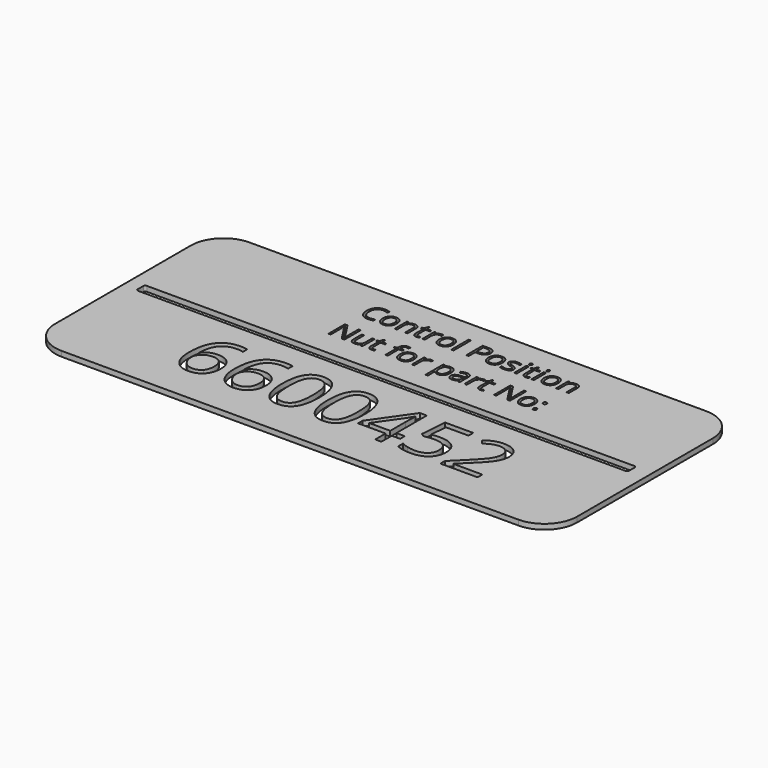
from build123d import *

# Parameters (mm, degrees)
F0_W     = 0.3558708372
F0_H     = 3.3344891736
F0_H_2   = 2.348473251
F1_DEPTH = 0.8


with BuildPart() as f1:
    # F0 (on Top) → F1 (new body)
    with BuildSketch(Plane.XY):
        with BuildLine():
            ThreePointArc((0, 5), (1.4644660941, 1.4644660941), (5, 0))
            Line((5, 0), (75, 0))
            ThreePointArc((75, 0), (78.5355339059, 1.4644660941), (80, 5))
            Line((80, 5), (80, 31))
            ThreePointArc((80, 31), (78.5355339059, 34.5355339059), (75, 36))
            Line((75, 36), (5, 36))
            ThreePointArc((5, 36), (1.4644660941, 34.5355339059), (0, 31))
            Line((0, 31), (0, 5))
        make_face()
        with BuildLine():
            add(Edge.make_bspline(
                [(17.8983092846, 6.4021890964), (17.1103991161, 7.4129138132), (17.1103991161, 9.2143931397)],
                knots=[0, 0, 0, 1, 1, 1], degree=2))
            add(Edge.make_bspline(
                [(17.1103991161, 9.2143931397), (17.1103991161, 11.7687011953), (18.1031090397, 13.0335293118)],
                knots=[0, 0, 0, 1, 1, 1], degree=2))
            add(Edge.make_bspline(
                [(18.1031090397, 13.0335293118), (19.0958189633, 14.2983574284), (21.0395203418, 14.2983574284)],
                knots=[0, 0, 0, 1, 1, 1], degree=2))
            add(Edge.make_bspline(
                [(21.0395203418, 14.2983574284), (21.7089121337, 14.2983574284), (22.0938598213, 14.1864760808)],
                knots=[0, 0, 0, 1, 1, 1], degree=2))
            Line((22.0938598213, 14.1864760808), (22.0938598213, 13.3388326503))
            add(Edge.make_bspline(
                [(22.0938598213, 13.3388326503), (21.6368529606, 13.4867435845), (21.050898106, 13.4867435845)],
                knots=[0, 0, 0, 1, 1, 1], degree=2))
            add(Edge.make_bspline(
                [(21.050898106, 13.4867435845), (19.6571219955, 13.4867435845), (18.9223080597, 12.6191890668)],
                knots=[0, 0, 0, 1, 1, 1], degree=2))
            add(Edge.make_bspline(
                [(18.9223080597, 12.6191890668), (18.1874941239, 11.751634549), (18.1173312449, 9.8894738136)],
                knots=[0, 0, 0, 1, 1, 1], degree=2))
            Line((18.1173312449, 9.8894738136), (18.1874941239, 9.8894738136))
            add(Edge.make_bspline(
                [(18.1874941239, 9.8894738136), (18.8398192695, 10.9096800006), (20.2506620262, 10.9096800006)],
                knots=[0, 0, 0, 1, 1, 1], degree=2))
            add(Edge.make_bspline(
                [(20.2506620262, 10.9096800006), (21.4187791474, 10.9096800006), (22.0910153803, 10.2042586223)],
                knots=[0, 0, 0, 1, 1, 1], degree=2))
            add(Edge.make_bspline(
                [(22.0910153803, 10.2042586223), (22.7632516132, 9.4988372439), (22.7632516132, 8.2908979481)],
                knots=[0, 0, 0, 1, 1, 1], degree=2))
            add(Edge.make_bspline(
                [(22.7632516132, 8.2908979481), (22.7632516132, 6.9388403062), (22.0255932363, 6.1651523429)],
                knots=[0, 0, 0, 1, 1, 1], degree=2))
            add(Edge.make_bspline(
                [(22.0255932363, 6.1651523429), (21.2879348595, 5.3914643795), (20.030691919, 5.3914643795)],
                knots=[0, 0, 0, 1, 1, 1], degree=2))
            add(Edge.make_bspline(
                [(20.030691919, 5.3914643795), (18.6862194532, 5.3914643795), (17.8983092846, 6.4021890964)],
                knots=[0, 0, 0, 1, 1, 1], degree=2))
        make_face(mode=Mode.SUBTRACT)
        with BuildLine():
            add(Edge.make_bspline(
                [(24.8368491326, 6.4021890964), (24.0489389641, 7.4129138132), (24.0489389641, 9.2143931397)],
                knots=[0, 0, 0, 1, 1, 1], degree=2))
            add(Edge.make_bspline(
                [(24.0489389641, 9.2143931397), (24.0489389641, 11.7687011953), (25.0416488877, 13.0335293118)],
                knots=[0, 0, 0, 1, 1, 1], degree=2))
            add(Edge.make_bspline(
                [(25.0416488877, 13.0335293118), (26.0343588113, 14.2983574284), (27.9780601898, 14.2983574284)],
                knots=[0, 0, 0, 1, 1, 1], degree=2))
            add(Edge.make_bspline(
                [(27.9780601898, 14.2983574284), (28.6474519817, 14.2983574284), (29.0323996693, 14.1864760808)],
                knots=[0, 0, 0, 1, 1, 1], degree=2))
            Line((29.0323996693, 14.1864760808), (29.0323996693, 13.3388326503))
            add(Edge.make_bspline(
                [(29.0323996693, 13.3388326503), (28.5753928086, 13.4867435845), (27.989437954, 13.4867435845)],
                knots=[0, 0, 0, 1, 1, 1], degree=2))
            add(Edge.make_bspline(
                [(27.989437954, 13.4867435845), (26.5956618435, 13.4867435845), (25.8608479077, 12.6191890668)],
                knots=[0, 0, 0, 1, 1, 1], degree=2))
            add(Edge.make_bspline(
                [(25.8608479077, 12.6191890668), (25.1260339719, 11.751634549), (25.0558710929, 9.8894738136)],
                knots=[0, 0, 0, 1, 1, 1], degree=2))
            Line((25.0558710929, 9.8894738136), (25.1260339719, 9.8894738136))
            add(Edge.make_bspline(
                [(25.1260339719, 9.8894738136), (25.7783591175, 10.9096800006), (27.1892018742, 10.9096800006)],
                knots=[0, 0, 0, 1, 1, 1], degree=2))
            add(Edge.make_bspline(
                [(27.1892018742, 10.9096800006), (28.3573189954, 10.9096800006), (29.0295552283, 10.2042586223)],
                knots=[0, 0, 0, 1, 1, 1], degree=2))
            add(Edge.make_bspline(
                [(29.0295552283, 10.2042586223), (29.7017914612, 9.4988372439), (29.7017914612, 8.2908979481)],
                knots=[0, 0, 0, 1, 1, 1], degree=2))
            add(Edge.make_bspline(
                [(29.7017914612, 8.2908979481), (29.7017914612, 6.9388403062), (28.9641330843, 6.1651523429)],
                knots=[0, 0, 0, 1, 1, 1], degree=2))
            add(Edge.make_bspline(
                [(28.9641330843, 6.1651523429), (28.2264747075, 5.3914643795), (26.969231767, 5.3914643795)],
                knots=[0, 0, 0, 1, 1, 1], degree=2))
            add(Edge.make_bspline(
                [(26.969231767, 5.3914643795), (25.6247593012, 5.3914643795), (24.8368491326, 6.4021890964)],
                knots=[0, 0, 0, 1, 1, 1], degree=2))
        make_face(mode=Mode.SUBTRACT)
        with BuildLine():
            add(Edge.make_bspline(
                [(35.8969840502, 13.1672180408), (36.628953545, 12.022804595), (36.628953545, 9.8553405211)],
                knots=[0, 0, 0, 1, 1, 1], degree=2))
            add(Edge.make_bspline(
                [(36.628953545, 9.8553405211), (36.628953545, 7.6082320981), (35.9206877256, 6.4998482388)],
                knots=[0, 0, 0, 1, 1, 1], degree=2))
            add(Edge.make_bspline(
                [(35.9206877256, 6.4998482388), (35.2124219062, 5.3914643795), (33.7541717987, 5.3914643795)],
                knots=[0, 0, 0, 1, 1, 1], degree=2))
            add(Edge.make_bspline(
                [(33.7541717987, 5.3914643795), (32.3566031002, 5.3914643795), (31.6274780465, 6.5263963552)],
                knots=[0, 0, 0, 1, 1, 1], degree=2))
            add(Edge.make_bspline(
                [(31.6274780465, 6.5263963552), (30.8983529928, 7.6613283309), (30.8983529928, 9.8553405211)],
                knots=[0, 0, 0, 1, 1, 1], degree=2))
            add(Edge.make_bspline(
                [(30.8983529928, 9.8553405211), (30.8983529928, 12.1176192964), (31.6037743711, 13.2146253915)],
                knots=[0, 0, 0, 1, 1, 1], degree=2))
            add(Edge.make_bspline(
                [(31.6037743711, 13.2146253915), (32.3091957495, 14.3116314866), (33.7541717987, 14.3116314866)],
                knots=[0, 0, 0, 1, 1, 1], degree=2))
            add(Edge.make_bspline(
                [(33.7541717987, 14.3116314866), (35.1650145555, 14.3116314866), (35.8969840502, 13.1672180408)],
                knots=[0, 0, 0, 1, 1, 1], degree=2))
        make_face(mode=Mode.SUBTRACT)
        with BuildLine():
            add(Edge.make_bspline(
                [(42.8355238982, 13.1672180408), (43.567493393, 12.022804595), (43.567493393, 9.8553405211)],
                knots=[0, 0, 0, 1, 1, 1], degree=2))
            add(Edge.make_bspline(
                [(43.567493393, 9.8553405211), (43.567493393, 7.6082320981), (42.8592275736, 6.4998482388)],
                knots=[0, 0, 0, 1, 1, 1], degree=2))
            add(Edge.make_bspline(
                [(42.8592275736, 6.4998482388), (42.1509617542, 5.3914643795), (40.6927116467, 5.3914643795)],
                knots=[0, 0, 0, 1, 1, 1], degree=2))
            add(Edge.make_bspline(
                [(40.6927116467, 5.3914643795), (39.2951429482, 5.3914643795), (38.5660178945, 6.5263963552)],
                knots=[0, 0, 0, 1, 1, 1], degree=2))
            add(Edge.make_bspline(
                [(38.5660178945, 6.5263963552), (37.8368928408, 7.6613283309), (37.8368928408, 9.8553405211)],
                knots=[0, 0, 0, 1, 1, 1], degree=2))
            add(Edge.make_bspline(
                [(37.8368928408, 9.8553405211), (37.8368928408, 12.1176192964), (38.5423142191, 13.2146253915)],
                knots=[0, 0, 0, 1, 1, 1], degree=2))
            add(Edge.make_bspline(
                [(38.5423142191, 13.2146253915), (39.2477355975, 14.3116314866), (40.6927116467, 14.3116314866)],
                knots=[0, 0, 0, 1, 1, 1], degree=2))
            add(Edge.make_bspline(
                [(40.6927116467, 14.3116314866), (42.1035544035, 14.3116314866), (42.8355238982, 13.1672180408)],
                knots=[0, 0, 0, 1, 1, 1], degree=2))
        make_face(mode=Mode.SUBTRACT)
        Polygon((50.8663291063, 8.3970904137), (50.8663291063, 7.5020396325), (49.5806417554, 7.5020396325), (49.5806417554, 5.5109309033), (48.6381836236, 5.5109309033), (48.6381836236, 7.5020396325), (44.4246182936, 7.5020396325), (44.4246182936, 8.3610608272), (48.5376800401, 14.2225056673), (49.5806417554, 14.2225056673), (49.5806417554, 8.3970904137), align=None, mode=Mode.SUBTRACT)
        with BuildLine():
            add(Edge.make_bspline(
                [(53.0527561205, 10.6669543651), (53.7335256765, 10.8034875351), (54.4105026444, 10.8034875351)],
                knots=[0, 0, 0, 1, 1, 1], degree=2))
            add(Edge.make_bspline(
                [(54.4105026444, 10.8034875351), (55.7796269325, 10.8034875351), (56.5646926601, 10.1246142731)],
                knots=[0, 0, 0, 1, 1, 1], degree=2))
            add(Edge.make_bspline(
                [(56.5646926601, 10.1246142731), (57.3497583876, 9.4457410111), (57.3497583876, 8.2662461258)],
                knots=[0, 0, 0, 1, 1, 1], degree=2))
            add(Edge.make_bspline(
                [(57.3497583876, 8.2662461258), (57.3497583876, 6.92177366), (56.493581634, 6.1566190197)],
                knots=[0, 0, 0, 1, 1, 1], degree=2))
            add(Edge.make_bspline(
                [(56.493581634, 6.1566190197), (55.6374048804, 5.3914643795), (54.1317474223, 5.3914643795)],
                knots=[0, 0, 0, 1, 1, 1], degree=2))
            add(Edge.make_bspline(
                [(54.1317474223, 5.3914643795), (52.6678084328, 5.3914643795), (51.8979130575, 5.8598490044)],
                knots=[0, 0, 0, 1, 1, 1], degree=2))
            Line((51.8979130575, 5.8598490044), (51.8979130575, 6.8079960183))
            add(Edge.make_bspline(
                [(51.8979130575, 6.8079960183), (52.3113051556, 6.5425148544), (52.9276007146, 6.3908113322)],
                knots=[0, 0, 0, 1, 1, 1], degree=2))
            add(Edge.make_bspline(
                [(52.9276007146, 6.3908113322), (53.5438962737, 6.23910781), (54.1431251865, 6.23910781)],
                knots=[0, 0, 0, 1, 1, 1], degree=2))
            add(Edge.make_bspline(
                [(54.1431251865, 6.23910781), (55.1860869018, 6.23910781), (55.7635084333, 6.7311961102)],
                knots=[0, 0, 0, 1, 1, 1], degree=2))
            add(Edge.make_bspline(
                [(55.7635084333, 6.7311961102), (56.3409299648, 7.2232844104), (56.3409299648, 8.1543647781)],
                knots=[0, 0, 0, 1, 1, 1], degree=2))
            add(Edge.make_bspline(
                [(56.3409299648, 8.1543647781), (56.3409299648, 9.9672218688), (54.1203696581, 9.9672218688)],
                knots=[0, 0, 0, 1, 1, 1], degree=2))
            add(Edge.make_bspline(
                [(54.1203696581, 9.9672218688), (53.5571703319, 9.9672218688), (52.6147122, 9.7946591122)],
                knots=[0, 0, 0, 1, 1, 1], degree=2))
            Line((52.6147122, 9.7946591122), (52.1046091065, 10.120821685))
            Line((52.1046091065, 10.120821685), (52.4307716793, 14.1750983166))
            Line((52.4307716793, 14.1750983166), (56.7391517106, 14.1750983166))
            Line((56.7391517106, 14.1750983166), (56.7391517106, 13.2686697713))
            Line((56.7391517106, 13.2686697713), (53.2727262277, 13.2686697713))
            Line((53.2727262277, 13.2686697713), (53.0527561205, 10.6669543651))
        make_face(mode=Mode.SUBTRACT)
        with BuildLine():
            Line((64.3357055863, 6.4230483307), (64.3357055863, 5.5109309033))
            Line((64.3357055863, 5.5109309033), (58.6411346206, 5.5109309033))
            Line((58.6411346206, 5.5109309033), (58.6411346206, 6.3585743337))
            Line((58.6411346206, 6.3585743337), (60.9223763361, 8.6511938134))
            add(Edge.make_bspline(
                [(60.9223763361, 8.6511938134), (61.9653380515, 9.7074295869), (62.2971895064, 10.1577994186)],
                knots=[0, 0, 0, 1, 1, 1], degree=2))
            add(Edge.make_bspline(
                [(62.2971895064, 10.1577994186), (62.6290409612, 10.6081692502), (62.7949666887, 11.0348354065)],
                knots=[0, 0, 0, 1, 1, 1], degree=2))
            add(Edge.make_bspline(
                [(62.7949666887, 11.0348354065), (62.9608924161, 11.4615015627), (62.9608924161, 11.952641716)],
                knots=[0, 0, 0, 1, 1, 1], degree=2))
            add(Edge.make_bspline(
                [(62.9608924161, 11.952641716), (62.9608924161, 12.6466853302), (62.5399151419, 13.0524922521)],
                knots=[0, 0, 0, 1, 1, 1], degree=2))
            add(Edge.make_bspline(
                [(62.5399151419, 13.0524922521), (62.1189378677, 13.4582991741), (61.3717980207, 13.4582991741)],
                knots=[0, 0, 0, 1, 1, 1], degree=2))
            add(Edge.make_bspline(
                [(61.3717980207, 13.4582991741), (60.8332505168, 13.4582991741), (60.3496955397, 13.2800475355)],
                knots=[0, 0, 0, 1, 1, 1], degree=2))
            add(Edge.make_bspline(
                [(60.3496955397, 13.2800475355), (59.8661405626, 13.1017958968), (59.2744968259, 12.633411272)],
                knots=[0, 0, 0, 1, 1, 1], degree=2))
            Line((59.2744968259, 12.633411272), (58.7530159683, 13.3028030638))
            add(Edge.make_bspline(
                [(58.7530159683, 13.3028030638), (59.9495774998, 14.2983574284), (61.3604202566, 14.2983574284)],
                knots=[0, 0, 0, 1, 1, 1], degree=2))
            add(Edge.make_bspline(
                [(61.3604202566, 14.2983574284), (62.5816336105, 14.2983574284), (63.2747290777, 13.6735285463)],
                knots=[0, 0, 0, 1, 1, 1], degree=2))
            add(Edge.make_bspline(
                [(63.2747290777, 13.6735285463), (63.9678245449, 13.0486996641), (63.9678245449, 11.9943601846)],
                knots=[0, 0, 0, 1, 1, 1], degree=2))
            add(Edge.make_bspline(
                [(63.9678245449, 11.9943601846), (63.9678245449, 11.1694722824), (63.5051288021, 10.3635473206)],
                knots=[0, 0, 0, 1, 1, 1], degree=2))
            add(Edge.make_bspline(
                [(63.5051288021, 10.3635473206), (63.0424330593, 9.5576223587), (61.7757086487, 8.3250312406)],
                knots=[0, 0, 0, 1, 1, 1], degree=2))
            Line((61.7757086487, 8.3250312406), (59.8794146208, 6.4704556814))
            Line((59.8794146208, 6.4704556814), (59.8794146208, 6.4230483307))
            Line((59.8794146208, 6.4230483307), (64.3357055863, 6.4230483307))
        make_face(mode=Mode.SUBTRACT)
        with BuildLine():
            ThreePointArc((2.1210229024, 19.2288067192), (2.2088908681, 19.4409387535), (2.4210229024, 19.5288067192))
            Line((2.4210229024, 19.5288067192), (77.1353295565, 19.5288067192))
            ThreePointArc((77.1353295565, 19.5288067192), (77.3474615908, 19.4409387535), (77.4353295565, 19.2288067192))
            Line((77.4353295565, 19.2288067192), (77.4353295565, 18.167911607))
            ThreePointArc((77.4353295565, 18.167911607), (77.3474615908, 17.9557795727), (77.1353295565, 17.867911607))
            Line((77.1353295565, 17.867911607), (2.4210229024, 17.867911607))
            ThreePointArc((2.4210229024, 17.867911607), (2.2088908681, 17.9557795727), (2.1210229024, 18.167911607))
            Line((2.1210229024, 18.167911607), (2.1210229024, 19.2288067192))
        make_face(mode=Mode.SUBTRACT)
        with BuildLine():
            Line((29.5978173932, 26.5573431885), (29.5978173932, 23.4244455874))
            Line((29.5978173932, 23.4244455874), (29.182291907, 23.4244455874))
            Line((29.182291907, 23.4244455874), (27.4701349121, 26.0533642573))
            Line((27.4701349121, 26.0533642573), (27.4529927716, 26.0533642573))
            add(Edge.make_bspline(
                [(27.4529927716, 26.0533642573), (27.4872770526, 25.5905264633), (27.4872770526, 25.2051711444)],
                knots=[0, 0, 0, 1, 1, 1], degree=2))
            Line((27.4872770526, 25.2051711444), (27.4872770526, 23.4244455874))
            Line((27.4872770526, 23.4244455874), (27.1506054128, 23.4244455874))
            Line((27.1506054128, 23.4244455874), (27.1506054128, 26.5573431885))
            Line((27.1506054128, 26.5573431885), (27.5620167853, 26.5573431885))
            Line((27.5620167853, 26.5573431885), (29.2700596665, 23.938709803))
            Line((29.2700596665, 23.938709803), (29.287201807, 23.938709803))
            add(Edge.make_bspline(
                [(29.287201807, 23.938709803), (29.2830876933, 23.9963073951), (29.2680026096, 24.3103514094)],
                knots=[0, 0, 0, 1, 1, 1], degree=2))
            add(Edge.make_bspline(
                [(29.2680026096, 24.3103514094), (29.252917526, 24.6243954237), (29.2570316397, 24.759475491)],
                knots=[0, 0, 0, 1, 1, 1], degree=2))
            Line((29.2570316397, 24.759475491), (29.2570316397, 26.5573431885))
            Line((29.2570316397, 26.5573431885), (29.5978173932, 26.5573431885))
        make_face(mode=Mode.SUBTRACT)
        with BuildLine():
            Line((30.3801846864, 25.7729188384), (30.7401696373, 25.7729188384))
            Line((30.7401696373, 25.7729188384), (30.7401696373, 24.2493253891))
            add(Edge.make_bspline(
                [(30.7401696373, 24.2493253891), (30.7401696373, 23.9620231141), (30.870792748, 23.8207718762)],
                knots=[0, 0, 0, 1, 1, 1], degree=2))
            add(Edge.make_bspline(
                [(30.870792748, 23.8207718762), (31.0014158588, 23.6795206383), (31.2798042208, 23.6795206383)],
                knots=[0, 0, 0, 1, 1, 1], degree=2))
            add(Edge.make_bspline(
                [(31.2798042208, 23.6795206383), (31.6487030848, 23.6795206383), (31.8187531187, 23.880769368)],
                knots=[0, 0, 0, 1, 1, 1], degree=2))
            add(Edge.make_bspline(
                [(31.8187531187, 23.880769368), (31.9888031526, 24.0820180977), (31.9888031526, 24.5386847211)],
                knots=[0, 0, 0, 1, 1, 1], degree=2))
            Line((31.9888031526, 24.5386847211), (31.9888031526, 25.7729188384))
            Line((31.9888031526, 25.7729188384), (32.3446739898, 25.7729188384))
            Line((32.3446739898, 25.7729188384), (32.3446739898, 23.4244455874))
            Line((32.3446739898, 23.4244455874), (32.0512005441, 23.4244455874))
            Line((32.0512005441, 23.4244455874), (31.9997741226, 23.7391752873))
            Line((31.9997741226, 23.7391752873), (31.9805749252, 23.7391752873))
            add(Edge.make_bspline(
                [(31.9805749252, 23.7391752873), (31.8715509115, 23.5656968253), (31.6775018808, 23.4734721093)],
                knots=[0, 0, 0, 1, 1, 1], degree=2))
            add(Edge.make_bspline(
                [(31.6775018808, 23.4734721093), (31.4834528502, 23.3812473933), (31.2345489698, 23.3812473933)],
                knots=[0, 0, 0, 1, 1, 1], degree=2))
            add(Edge.make_bspline(
                [(31.2345489698, 23.3812473933), (30.8059954569, 23.3812473933), (30.5930900717, 23.5848960227)],
                knots=[0, 0, 0, 1, 1, 1], degree=2))
            add(Edge.make_bspline(
                [(30.5930900717, 23.5848960227), (30.3801846864, 23.788544652), (30.3801846864, 24.2362973624)],
                knots=[0, 0, 0, 1, 1, 1], degree=2))
            Line((30.3801846864, 24.2362973624), (30.3801846864, 25.7729188384))
        make_face(mode=Mode.SUBTRACT)
        with BuildLine():
            add(Edge.make_bspline(
                [(39.0119381229, 25.488016463), (39.3023259833, 25.1599158935), (39.3023259833, 24.6010821126)],
                knots=[0, 0, 0, 1, 1, 1], degree=2))
            add(Edge.make_bspline(
                [(39.3023259833, 24.6010821126), (39.3023259833, 24.0264775624), (39.0133094941, 23.7038624779)],
                knots=[0, 0, 0, 1, 1, 1], degree=2))
            add(Edge.make_bspline(
                [(39.0133094941, 23.7038624779), (38.724293005, 23.3812473933), (38.2141429032, 23.3812473933)],
                knots=[0, 0, 0, 1, 1, 1], degree=2))
            add(Edge.make_bspline(
                [(38.2141429032, 23.3812473933), (37.8987275176, 23.3812473933), (37.6546234367, 23.5293554874)],
                knots=[0, 0, 0, 1, 1, 1], degree=2))
            add(Edge.make_bspline(
                [(37.6546234367, 23.5293554874), (37.4105193557, 23.6774635815), (37.2774963453, 23.9537948866)],
                knots=[0, 0, 0, 1, 1, 1], degree=2))
            add(Edge.make_bspline(
                [(37.2774963453, 23.9537948866), (37.1444733348, 24.2301261918), (37.1444733348, 24.6010821126)],
                knots=[0, 0, 0, 1, 1, 1], degree=2))
            add(Edge.make_bspline(
                [(37.1444733348, 24.6010821126), (37.1444733348, 25.1750009771), (37.4317756099, 25.4955590048)],
                knots=[0, 0, 0, 1, 1, 1], degree=2))
            add(Edge.make_bspline(
                [(37.4317756099, 25.4955590048), (37.719077885, 25.8161170325), (38.2292279868, 25.8161170325)],
                knots=[0, 0, 0, 1, 1, 1], degree=2))
            add(Edge.make_bspline(
                [(38.2292279868, 25.8161170325), (38.7215502625, 25.8161170325), (39.0119381229, 25.488016463)],
                knots=[0, 0, 0, 1, 1, 1], degree=2))
        make_face(mode=Mode.SUBTRACT)
        with BuildLine():
            add(Edge.make_bspline(
                [(33.580965164, 23.7888874948), (33.6817609502, 23.6754065246), (33.8572964691, 23.6754065246)],
                knots=[0, 0, 0, 1, 1, 1], degree=2))
            add(Edge.make_bspline(
                [(33.8572964691, 23.6754065246), (33.9519210848, 23.6754065246), (34.0396888442, 23.689120237)],
                knots=[0, 0, 0, 1, 1, 1], degree=2))
            add(Edge.make_bspline(
                [(34.0396888442, 23.689120237), (34.1274566037, 23.7028339494), (34.1788830252, 23.7179190331)],
                knots=[0, 0, 0, 1, 1, 1], degree=2))
            Line((34.1788830252, 23.7179190331), (34.1788830252, 23.4457018417))
            add(Edge.make_bspline(
                [(34.1788830252, 23.4457018417), (34.1212854331, 23.4182744168), (34.0088329913, 23.3997609051)],
                knots=[0, 0, 0, 1, 1, 1], degree=2))
            add(Edge.make_bspline(
                [(34.0088329913, 23.3997609051), (33.8963805495, 23.3812473933), (33.8058700476, 23.3812473933)],
                knots=[0, 0, 0, 1, 1, 1], degree=2))
            add(Edge.make_bspline(
                [(33.8058700476, 23.3812473933), (33.1249842262, 23.3812473933), (33.1249842262, 24.0991602382)],
                knots=[0, 0, 0, 1, 1, 1], degree=2))
            Line((33.1249842262, 24.0991602382), (33.1249842262, 25.4965875332))
            Line((33.1249842262, 25.4965875332), (32.7883125864, 25.4965875332))
            Line((32.7883125864, 25.4965875332), (32.7883125864, 25.6680089384))
            Line((32.7883125864, 25.6680089384), (33.1249842262, 25.8161170325))
            Line((33.1249842262, 25.8161170325), (33.2744636915, 26.3173532212))
            Line((33.2744636915, 26.3173532212), (33.4801693777, 26.3173532212))
            Line((33.4801693777, 26.3173532212), (33.4801693777, 25.7729188384))
            Line((33.4801693777, 25.7729188384), (34.1617408847, 25.7729188384))
            Line((34.1617408847, 25.7729188384), (34.1617408847, 25.4965875332))
            Line((34.1617408847, 25.4965875332), (33.4801693777, 25.4965875332))
            Line((33.4801693777, 25.4965875332), (33.4801693777, 24.1142453219))
            add(Edge.make_bspline(
                [(33.4801693777, 24.1142453219), (33.4801693777, 23.9023684651), (33.580965164, 23.7888874948)],
                knots=[0, 0, 0, 1, 1, 1], degree=2))
        make_face(mode=Mode.SUBTRACT)
        with BuildLine():
            Line((36.8468857755, 25.7729188384), (36.8468857755, 25.4965875332))
            Line((36.8468857755, 25.4965875332), (36.2489679142, 25.4965875332))
            Line((36.2489679142, 25.4965875332), (36.2489679142, 23.4244455874))
            Line((36.2489679142, 23.4244455874), (35.893097077, 23.4244455874))
            Line((35.893097077, 23.4244455874), (35.893097077, 25.4965875332))
            Line((35.893097077, 25.4965875332), (35.4734574771, 25.4965875332))
            Line((35.4734574771, 25.4965875332), (35.4734574771, 25.6570379685))
            Line((35.4734574771, 25.6570379685), (35.893097077, 25.7859468652))
            Line((35.893097077, 25.7859468652), (35.893097077, 25.9162271331))
            add(Edge.make_bspline(
                [(35.893097077, 25.9162271331), (35.893097077, 26.7822480721), (36.6494083167, 26.7822480721)],
                knots=[0, 0, 0, 1, 1, 1], degree=2))
            add(Edge.make_bspline(
                [(36.6494083167, 26.7822480721), (36.8359148055, 26.7822480721), (37.0868757427, 26.7075083394)],
                knots=[0, 0, 0, 1, 1, 1], degree=2))
            Line((37.0868757427, 26.7075083394), (36.9943081839, 26.4222631212))
            add(Edge.make_bspline(
                [(36.9943081839, 26.4222631212), (36.7886024977, 26.4887746264), (36.6432371461, 26.4887746264)],
                knots=[0, 0, 0, 1, 1, 1], degree=2))
            add(Edge.make_bspline(
                [(36.6432371461, 26.4887746264), (36.4416455736, 26.4887746264), (36.3453067439, 26.3547230876)],
                knots=[0, 0, 0, 1, 1, 1], degree=2))
            add(Edge.make_bspline(
                [(36.3453067439, 26.3547230876), (36.2489679142, 26.2206715487), (36.2489679142, 25.9251410462)],
                knots=[0, 0, 0, 1, 1, 1], degree=2))
            Line((36.2489679142, 25.9251410462), (36.2489679142, 25.7729188384))
            Line((36.2489679142, 25.7729188384), (36.8468857755, 25.7729188384))
        make_face(mode=Mode.SUBTRACT)
        with BuildLine():
            add(Edge.make_bspline(
                [(29.2035481613, 32.0777981209), (28.8476773241, 32.2444197268), (28.491806487, 32.2444197268)],
                knots=[0, 0, 0, 1, 1, 1], degree=2))
            add(Edge.make_bspline(
                [(28.491806487, 32.2444197268), (27.9754852145, 32.2444197268), (27.6765262839, 31.900548388)],
                knots=[0, 0, 0, 1, 1, 1], degree=2))
            add(Edge.make_bspline(
                [(27.6765262839, 31.900548388), (27.3775673533, 31.5566770492), (27.3775673533, 30.9587591879)],
                knots=[0, 0, 0, 1, 1, 1], degree=2))
            add(Edge.make_bspline(
                [(27.3775673533, 30.9587591879), (27.3775673533, 30.3443848717), (27.6658981568, 30.0087417604)],
                knots=[0, 0, 0, 1, 1, 1], degree=2))
            add(Edge.make_bspline(
                [(27.6658981568, 30.0087417604), (27.9542289603, 29.6730986491), (28.4876923732, 29.6730986491)],
                knots=[0, 0, 0, 1, 1, 1], degree=2))
            add(Edge.make_bspline(
                [(28.4876923732, 29.6730986491), (28.8154500999, 29.6730986491), (29.2357753854, 29.7910365758)],
                knots=[0, 0, 0, 1, 1, 1], degree=2))
            Line((29.2357753854, 29.7910365758), (29.2357753854, 29.4721927622))
            add(Edge.make_bspline(
                [(29.2357753854, 29.4721927622), (28.9100747156, 29.3494550361), (28.4321518379, 29.3494550361)],
                knots=[0, 0, 0, 1, 1, 1], degree=2))
            add(Edge.make_bspline(
                [(28.4321518379, 29.3494550361), (27.7402950466, 29.3494550361), (27.3641964837, 29.7697803216)],
                knots=[0, 0, 0, 1, 1, 1], degree=2))
            add(Edge.make_bspline(
                [(27.3641964837, 29.7697803216), (26.9880979207, 30.1901056071), (26.9880979207, 30.9635589873)],
                knots=[0, 0, 0, 1, 1, 1], degree=2))
            add(Edge.make_bspline(
                [(26.9880979207, 30.9635589873), (26.9880979207, 31.4476530355), (27.1691189246, 31.8117521001)],
                knots=[0, 0, 0, 1, 1, 1], degree=2))
            add(Edge.make_bspline(
                [(27.1691189246, 31.8117521001), (27.3501399285, 32.1758511647), (27.6919542104, 32.3729857807)],
                knots=[0, 0, 0, 1, 1, 1], degree=2))
            add(Edge.make_bspline(
                [(27.6919542104, 32.3729857807), (28.0337684923, 32.5701203966), (28.4966062863, 32.5701203966)],
                knots=[0, 0, 0, 1, 1, 1], degree=2))
            add(Edge.make_bspline(
                [(28.4966062863, 32.5701203966), (28.988928562, 32.5701203966), (29.3578274259, 32.390470764)],
                knots=[0, 0, 0, 1, 1, 1], degree=2))
            Line((29.3578274259, 32.390470764), (29.2035481613, 32.0777981209))
        make_face(mode=Mode.SUBTRACT)
        with BuildLine():
            add(Edge.make_bspline(
                [(31.6024193054, 31.4562241057), (31.8928071657, 31.1281235362), (31.8928071657, 30.5692897553)],
                knots=[0, 0, 0, 1, 1, 1], degree=2))
            add(Edge.make_bspline(
                [(31.8928071657, 30.5692897553), (31.8928071657, 29.9946852052), (31.6037906766, 29.6720701206)],
                knots=[0, 0, 0, 1, 1, 1], degree=2))
            add(Edge.make_bspline(
                [(31.6037906766, 29.6720701206), (31.3147741875, 29.3494550361), (30.8046240856, 29.3494550361)],
                knots=[0, 0, 0, 1, 1, 1], degree=2))
            add(Edge.make_bspline(
                [(30.8046240856, 29.3494550361), (30.4892087001, 29.3494550361), (30.2451046191, 29.4975631302)],
                knots=[0, 0, 0, 1, 1, 1], degree=2))
            add(Edge.make_bspline(
                [(30.2451046191, 29.4975631302), (30.0010005382, 29.6456712242), (29.8679775277, 29.9220025294)],
                knots=[0, 0, 0, 1, 1, 1], degree=2))
            add(Edge.make_bspline(
                [(29.8679775277, 29.9220025294), (29.7349545173, 30.1983338345), (29.7349545173, 30.5692897553)],
                knots=[0, 0, 0, 1, 1, 1], degree=2))
            add(Edge.make_bspline(
                [(29.7349545173, 30.5692897553), (29.7349545173, 31.1432086199), (30.0222567924, 31.4637666476)],
                knots=[0, 0, 0, 1, 1, 1], degree=2))
            add(Edge.make_bspline(
                [(30.0222567924, 31.4637666476), (30.3095590675, 31.7843246753), (30.8197091693, 31.7843246753)],
                knots=[0, 0, 0, 1, 1, 1], degree=2))
            add(Edge.make_bspline(
                [(30.8197091693, 31.7843246753), (31.312031445, 31.7843246753), (31.6024193054, 31.4562241057)],
                knots=[0, 0, 0, 1, 1, 1], degree=2))
        make_face(mode=Mode.SUBTRACT)
        with BuildLine():
            Line((34.4798990127, 29.3926532302), (34.1240281756, 29.3926532302))
            Line((34.1240281756, 29.3926532302), (34.1240281756, 30.9121325657))
            add(Edge.make_bspline(
                [(34.1240281756, 30.9121325657), (34.1240281756, 31.1987491552), (33.9934050648, 31.3403432358)],
                knots=[0, 0, 0, 1, 1, 1], degree=2))
            add(Edge.make_bspline(
                [(33.9934050648, 31.3403432358), (33.8627819541, 31.4819373165), (33.5837079064, 31.4819373165)],
                knots=[0, 0, 0, 1, 1, 1], degree=2))
            add(Edge.make_bspline(
                [(33.5837079064, 31.4819373165), (33.2154947281, 31.4819373165), (33.0440733229, 31.2827456437)],
                knots=[0, 0, 0, 1, 1, 1], degree=2))
            add(Edge.make_bspline(
                [(33.0440733229, 31.2827456437), (32.8726519177, 31.0835539709), (32.8726519177, 30.6248302906)],
                knots=[0, 0, 0, 1, 1, 1], degree=2))
            Line((32.8726519177, 30.6248302906), (32.8726519177, 29.3926532302))
            Line((32.8726519177, 29.3926532302), (32.5167810806, 29.3926532302))
            Line((32.5167810806, 29.3926532302), (32.5167810806, 31.7411264812))
            Line((32.5167810806, 31.7411264812), (32.8061404125, 31.7411264812))
            Line((32.8061404125, 31.7411264812), (32.8637380047, 31.419539925))
            Line((32.8637380047, 31.419539925), (32.8808801452, 31.419539925))
            add(Edge.make_bspline(
                [(32.8808801452, 31.419539925), (32.9905898445, 31.5930183871), (33.1877244605, 31.6886715312)],
                knots=[0, 0, 0, 1, 1, 1], degree=2))
            add(Edge.make_bspline(
                [(33.1877244605, 31.6886715312), (33.3848590764, 31.7843246753), (33.6269061005, 31.7843246753)],
                knots=[0, 0, 0, 1, 1, 1], degree=2))
            add(Edge.make_bspline(
                [(33.6269061005, 31.7843246753), (34.0513454998, 31.7843246753), (34.2656222562, 31.5796475175)],
                knots=[0, 0, 0, 1, 1, 1], degree=2))
            add(Edge.make_bspline(
                [(34.2656222562, 31.5796475175), (34.4798990127, 31.3749703597), (34.4798990127, 30.9244749069)],
                knots=[0, 0, 0, 1, 1, 1], degree=2))
            Line((34.4798990127, 30.9244749069), (34.4798990127, 29.3926532302))
        make_face(mode=Mode.SUBTRACT)
        with BuildLine():
            add(Edge.make_bspline(
                [(35.6921911902, 29.7570951376), (35.7929869764, 29.6436141674), (35.9685224953, 29.6436141674)],
                knots=[0, 0, 0, 1, 1, 1], degree=2))
            add(Edge.make_bspline(
                [(35.9685224953, 29.6436141674), (36.063147111, 29.6436141674), (36.1509148704, 29.6573278798)],
                knots=[0, 0, 0, 1, 1, 1], degree=2))
            add(Edge.make_bspline(
                [(36.1509148704, 29.6573278798), (36.2386826299, 29.6710415922), (36.2901090514, 29.6861266759)],
                knots=[0, 0, 0, 1, 1, 1], degree=2))
            Line((36.2901090514, 29.6861266759), (36.2901090514, 29.4139094844))
            add(Edge.make_bspline(
                [(36.2901090514, 29.4139094844), (36.2325114593, 29.3864820596), (36.1200590175, 29.3679685478)],
                knots=[0, 0, 0, 1, 1, 1], degree=2))
            add(Edge.make_bspline(
                [(36.1200590175, 29.3679685478), (36.0076065757, 29.3494550361), (35.9170960738, 29.3494550361)],
                knots=[0, 0, 0, 1, 1, 1], degree=2))
            add(Edge.make_bspline(
                [(35.9170960738, 29.3494550361), (35.2362102524, 29.3494550361), (35.2362102524, 30.067367881)],
                knots=[0, 0, 0, 1, 1, 1], degree=2))
            Line((35.2362102524, 30.067367881), (35.2362102524, 31.464795176))
            Line((35.2362102524, 31.464795176), (34.8995386126, 31.464795176))
            Line((34.8995386126, 31.464795176), (34.8995386126, 31.6362165812))
            Line((34.8995386126, 31.6362165812), (35.2362102524, 31.7843246753))
            Line((35.2362102524, 31.7843246753), (35.3856897177, 32.285560864))
            Line((35.3856897177, 32.285560864), (35.5913954039, 32.285560864))
            Line((35.5913954039, 32.285560864), (35.5913954039, 31.7411264812))
            Line((35.5913954039, 31.7411264812), (36.2729669109, 31.7411264812))
            Line((36.2729669109, 31.7411264812), (36.2729669109, 31.464795176))
            Line((36.2729669109, 31.464795176), (35.5913954039, 31.464795176))
            Line((35.5913954039, 31.464795176), (35.5913954039, 30.0824529646))
            add(Edge.make_bspline(
                [(35.5913954039, 30.0824529646), (35.5913954039, 29.8705761078), (35.6921911902, 29.7570951376)],
                knots=[0, 0, 0, 1, 1, 1], degree=2))
        make_face(mode=Mode.SUBTRACT)
        with BuildLine():
            add(Edge.make_bspline(
                [(37.4256044393, 31.6598727351), (37.6100538713, 31.7843246753), (37.8308446412, 31.7843246753)],
                knots=[0, 0, 0, 1, 1, 1], degree=2))
            add(Edge.make_bspline(
                [(37.8308446412, 31.7843246753), (37.9871809627, 31.7843246753), (38.1112900601, 31.7582686217)],
                knots=[0, 0, 0, 1, 1, 1], degree=2))
            Line((38.1112900601, 31.7582686217), (38.0619206954, 31.4284538381))
            add(Edge.make_bspline(
                [(38.0619206954, 31.4284538381), (37.9165553438, 31.4606810623), (37.8047885876, 31.4606810623)],
                knots=[0, 0, 0, 1, 1, 1], degree=2))
            add(Edge.make_bspline(
                [(37.8047885876, 31.4606810623), (37.5195433694, 31.4606810623), (37.3172661113, 31.2292621653)],
                knots=[0, 0, 0, 1, 1, 1], degree=2))
            add(Edge.make_bspline(
                [(37.3172661113, 31.2292621653), (37.1149888532, 30.9978432683), (37.1149888532, 30.6529434011)],
                knots=[0, 0, 0, 1, 1, 1], degree=2))
            Line((37.1149888532, 30.6529434011), (37.1149888532, 29.3926532302))
            Line((37.1149888532, 29.3926532302), (36.759118016, 29.3926532302))
            Line((36.759118016, 29.3926532302), (36.759118016, 31.7411264812))
            Line((36.759118016, 31.7411264812), (37.0525914617, 31.7411264812))
            Line((37.0525914617, 31.7411264812), (37.0937325989, 31.3064017976))
            Line((37.0937325989, 31.3064017976), (37.1108747394, 31.3064017976))
            add(Edge.make_bspline(
                [(37.1108747394, 31.3064017976), (37.2411550074, 31.5354207949), (37.4256044393, 31.6598727351)],
                knots=[0, 0, 0, 1, 1, 1], degree=2))
        make_face(mode=Mode.SUBTRACT)
        with BuildLine():
            add(Edge.make_bspline(
                [(40.2873133774, 31.4562241057), (40.5777012378, 31.1281235362), (40.5777012378, 30.5692897553)],
                knots=[0, 0, 0, 1, 1, 1], degree=2))
            add(Edge.make_bspline(
                [(40.5777012378, 30.5692897553), (40.5777012378, 29.9946852052), (40.2886847487, 29.6720701206)],
                knots=[0, 0, 0, 1, 1, 1], degree=2))
            add(Edge.make_bspline(
                [(40.2886847487, 29.6720701206), (39.9996682595, 29.3494550361), (39.4895181577, 29.3494550361)],
                knots=[0, 0, 0, 1, 1, 1], degree=2))
            add(Edge.make_bspline(
                [(39.4895181577, 29.3494550361), (39.1741027722, 29.3494550361), (38.9299986912, 29.4975631302)],
                knots=[0, 0, 0, 1, 1, 1], degree=2))
            add(Edge.make_bspline(
                [(38.9299986912, 29.4975631302), (38.6858946102, 29.6456712242), (38.5528715998, 29.9220025294)],
                knots=[0, 0, 0, 1, 1, 1], degree=2))
            add(Edge.make_bspline(
                [(38.5528715998, 29.9220025294), (38.4198485894, 30.1983338345), (38.4198485894, 30.5692897553)],
                knots=[0, 0, 0, 1, 1, 1], degree=2))
            add(Edge.make_bspline(
                [(38.4198485894, 30.5692897553), (38.4198485894, 31.1432086199), (38.7071508645, 31.4637666476)],
                knots=[0, 0, 0, 1, 1, 1], degree=2))
            add(Edge.make_bspline(
                [(38.7071508645, 31.4637666476), (38.9944531396, 31.7843246753), (39.5046032414, 31.7843246753)],
                knots=[0, 0, 0, 1, 1, 1], degree=2))
            add(Edge.make_bspline(
                [(39.5046032414, 31.7843246753), (39.9969255171, 31.7843246753), (40.2873133774, 31.4562241057)],
                knots=[0, 0, 0, 1, 1, 1], degree=2))
        make_face(mode=Mode.SUBTRACT)
        with BuildLine():
            add(Edge.make_bspline(
                [(40.5927863215, 25.6916650923), (40.7772357534, 25.8161170325), (40.9980265233, 25.8161170325)],
                knots=[0, 0, 0, 1, 1, 1], degree=2))
            add(Edge.make_bspline(
                [(40.9980265233, 25.8161170325), (41.1543628448, 25.8161170325), (41.2784719422, 25.7900609789)],
                knots=[0, 0, 0, 1, 1, 1], degree=2))
            Line((41.2784719422, 25.7900609789), (41.2291025775, 25.4602461953))
            add(Edge.make_bspline(
                [(41.2291025775, 25.4602461953), (41.0837372259, 25.4924734195), (40.9719704697, 25.4924734195)],
                knots=[0, 0, 0, 1, 1, 1], degree=2))
            add(Edge.make_bspline(
                [(40.9719704697, 25.4924734195), (40.6867252515, 25.4924734195), (40.4844479934, 25.2610545225)],
                knots=[0, 0, 0, 1, 1, 1], degree=2))
            add(Edge.make_bspline(
                [(40.4844479934, 25.2610545225), (40.2821707353, 25.0296356255), (40.2821707353, 24.6847357583)],
                knots=[0, 0, 0, 1, 1, 1], degree=2))
            Line((40.2821707353, 24.6847357583), (40.2821707353, 23.4244455874))
            Line((40.2821707353, 23.4244455874), (39.9262998981, 23.4244455874))
            Line((39.9262998981, 23.4244455874), (39.9262998981, 25.7729188384))
            Line((39.9262998981, 25.7729188384), (40.2197733438, 25.7729188384))
            Line((40.2197733438, 25.7729188384), (40.260914481, 25.3381941549))
            Line((40.260914481, 25.3381941549), (40.2780566216, 25.3381941549))
            add(Edge.make_bspline(
                [(40.2780566216, 25.3381941549), (40.4083368895, 25.5672131522), (40.5927863215, 25.6916650923)],
                knots=[0, 0, 0, 1, 1, 1], degree=2))
        make_face(mode=Mode.SUBTRACT)
        with BuildLine():
            add(Edge.make_bspline(
                [(44.6681588082, 23.701805421), (44.409998172, 23.3812473933), (43.9512744918, 23.3812473933)],
                knots=[0, 0, 0, 1, 1, 1], degree=2))
            add(Edge.make_bspline(
                [(43.9512744918, 23.3812473933), (43.7215698088, 23.3812473933), (43.5319777347, 23.4659295675)],
                knots=[0, 0, 0, 1, 1, 1], degree=2))
            add(Edge.make_bspline(
                [(43.5319777347, 23.4659295675), (43.3423856606, 23.5506117416), (43.2141624495, 23.7268329462)],
                knots=[0, 0, 0, 1, 1, 1], degree=2))
            Line((43.2141624495, 23.7268329462), (43.1881063959, 23.7268329462))
            add(Edge.make_bspline(
                [(43.1881063959, 23.7268329462), (43.2141624495, 23.5211272599), (43.2141624495, 23.336677828)],
                knots=[0, 0, 0, 1, 1, 1], degree=2))
            Line((43.2141624495, 23.336677828), (43.2141624495, 22.3698611027))
            Line((43.2141624495, 22.3698611027), (42.8582916123, 22.3698611027))
            Line((42.8582916123, 22.3698611027), (42.8582916123, 25.7729188384))
            Line((42.8582916123, 25.7729188384), (43.1476509443, 25.7729188384))
            Line((43.1476509443, 25.7729188384), (43.197020309, 25.4513322823))
            Line((43.197020309, 25.4513322823), (43.2141624495, 25.4513322823))
            add(Edge.make_bspline(
                [(43.2141624495, 25.4513322823), (43.3512995736, 25.6446956273), (43.5333491059, 25.7304063299)],
                knots=[0, 0, 0, 1, 1, 1], degree=2))
            add(Edge.make_bspline(
                [(43.5333491059, 25.7304063299), (43.7153986382, 25.8161170325), (43.9512744918, 25.8161170325)],
                knots=[0, 0, 0, 1, 1, 1], degree=2))
            add(Edge.make_bspline(
                [(43.9512744918, 25.8161170325), (44.4182263995, 25.8161170325), (44.6722729219, 25.4965875332)],
                knots=[0, 0, 0, 1, 1, 1], degree=2))
            add(Edge.make_bspline(
                [(44.6722729219, 25.4965875332), (44.9263194444, 25.177058034), (44.9263194444, 24.6010821126)],
                knots=[0, 0, 0, 1, 1, 1], degree=2))
            add(Edge.make_bspline(
                [(44.9263194444, 24.6010821126), (44.9263194444, 24.0223634487), (44.6681588082, 23.701805421)],
                knots=[0, 0, 0, 1, 1, 1], degree=2))
        make_face(mode=Mode.SUBTRACT)
        with BuildLine():
            Line((47.255593498, 23.4244455874), (46.991604534, 23.4244455874))
            Line((46.991604534, 23.4244455874), (46.9209789151, 23.7590601703))
            Line((46.9209789151, 23.7590601703), (46.9038367746, 23.7590601703))
            add(Edge.make_bspline(
                [(46.9038367746, 23.7590601703), (46.7283012557, 23.5382694005), (46.5537942652, 23.4597583969)],
                knots=[0, 0, 0, 1, 1, 1], degree=2))
            add(Edge.make_bspline(
                [(46.5537942652, 23.4597583969), (46.3792872747, 23.3812473933), (46.1173553676, 23.3812473933)],
                knots=[0, 0, 0, 1, 1, 1], degree=2))
            add(Edge.make_bspline(
                [(46.1173553676, 23.3812473933), (45.7683413867, 23.3812473933), (45.5701782423, 23.5615827116)],
                knots=[0, 0, 0, 1, 1, 1], degree=2))
            add(Edge.make_bspline(
                [(45.5701782423, 23.5615827116), (45.3720150979, 23.7419180298), (45.3720150979, 24.0737898702)],
                knots=[0, 0, 0, 1, 1, 1], degree=2))
            add(Edge.make_bspline(
                [(45.3720150979, 24.0737898702), (45.3720150979, 24.7848458589), (46.5095675427, 24.81913014)],
                knots=[0, 0, 0, 1, 1, 1], degree=2))
            Line((46.5095675427, 24.81913014), (46.9079508883, 24.8321581668))
            Line((46.9079508883, 24.8321581668), (46.9079508883, 24.978209204))
            add(Edge.make_bspline(
                [(46.9079508883, 24.978209204), (46.9079508883, 25.2545405091), (46.7893272759, 25.3861921483)],
                knots=[0, 0, 0, 1, 1, 1], degree=2))
            add(Edge.make_bspline(
                [(46.7893272759, 25.3861921483), (46.6707036635, 25.5178437875), (46.4087717564, 25.5178437875)],
                knots=[0, 0, 0, 1, 1, 1], degree=2))
            add(Edge.make_bspline(
                [(46.4087717564, 25.5178437875), (46.1152983108, 25.5178437875), (45.7450280756, 25.3381941549)],
                knots=[0, 0, 0, 1, 1, 1], degree=2))
            Line((45.7450280756, 25.3381941549), (45.6353183763, 25.6104113463))
            add(Edge.make_bspline(
                [(45.6353183763, 25.6104113463), (45.8087968383, 25.7043502763), (46.0155310529, 25.7578337547)],
                knots=[0, 0, 0, 1, 1, 1], degree=2))
            add(Edge.make_bspline(
                [(46.0155310529, 25.7578337547), (46.2222652676, 25.8113172331), (46.4307136963, 25.8113172331)],
                knots=[0, 0, 0, 1, 1, 1], degree=2))
            add(Edge.make_bspline(
                [(46.4307136963, 25.8113172331), (46.8503532962, 25.8113172331), (47.0529733971, 25.6251535871)],
                knots=[0, 0, 0, 1, 1, 1], degree=2))
            add(Edge.make_bspline(
                [(47.0529733971, 25.6251535871), (47.255593498, 25.4389899411), (47.255593498, 25.0275785687)],
                knots=[0, 0, 0, 1, 1, 1], degree=2))
            Line((47.255593498, 25.0275785687), (47.255593498, 23.4244455874))
        make_face(mode=Mode.SUBTRACT)
        with BuildLine():
            add(Edge.make_bspline(
                [(48.6543921643, 25.6916650923), (48.8388415963, 25.8161170325), (49.0596323661, 25.8161170325)],
                knots=[0, 0, 0, 1, 1, 1], degree=2))
            add(Edge.make_bspline(
                [(49.0596323661, 25.8161170325), (49.2159686877, 25.8161170325), (49.340077785, 25.7900609789)],
                knots=[0, 0, 0, 1, 1, 1], degree=2))
            Line((49.340077785, 25.7900609789), (49.2907084203, 25.4602461953))
            add(Edge.make_bspline(
                [(49.2907084203, 25.4602461953), (49.1453430687, 25.4924734195), (49.0335763126, 25.4924734195)],
                knots=[0, 0, 0, 1, 1, 1], degree=2))
            add(Edge.make_bspline(
                [(49.0335763126, 25.4924734195), (48.7483310943, 25.4924734195), (48.5460538362, 25.2610545225)],
                knots=[0, 0, 0, 1, 1, 1], degree=2))
            add(Edge.make_bspline(
                [(48.5460538362, 25.2610545225), (48.3437765781, 25.0296356255), (48.3437765781, 24.6847357583)],
                knots=[0, 0, 0, 1, 1, 1], degree=2))
            Line((48.3437765781, 24.6847357583), (48.3437765781, 23.4244455874))
            Line((48.3437765781, 23.4244455874), (47.987905741, 23.4244455874))
            Line((47.987905741, 23.4244455874), (47.987905741, 25.7729188384))
            Line((47.987905741, 25.7729188384), (48.2813791866, 25.7729188384))
            Line((48.2813791866, 25.7729188384), (48.3225203239, 25.3381941549))
            Line((48.3225203239, 25.3381941549), (48.3396624644, 25.3381941549))
            add(Edge.make_bspline(
                [(48.3396624644, 25.3381941549), (48.4699427323, 25.5672131522), (48.6543921643, 25.6916650923)],
                knots=[0, 0, 0, 1, 1, 1], degree=2))
        make_face(mode=Mode.SUBTRACT)
        with BuildLine():
            add(Edge.make_bspline(
                [(57.5137932268, 25.488016463), (57.8041810872, 25.1599158935), (57.8041810872, 24.6010821126)],
                knots=[0, 0, 0, 1, 1, 1], degree=2))
            add(Edge.make_bspline(
                [(57.8041810872, 24.6010821126), (57.8041810872, 24.0264775624), (57.5151645981, 23.7038624779)],
                knots=[0, 0, 0, 1, 1, 1], degree=2))
            add(Edge.make_bspline(
                [(57.5151645981, 23.7038624779), (57.2261481089, 23.3812473933), (56.7159980071, 23.3812473933)],
                knots=[0, 0, 0, 1, 1, 1], degree=2))
            add(Edge.make_bspline(
                [(56.7159980071, 23.3812473933), (56.4005826216, 23.3812473933), (56.1564785406, 23.5293554874)],
                knots=[0, 0, 0, 1, 1, 1], degree=2))
            add(Edge.make_bspline(
                [(56.1564785406, 23.5293554874), (55.9123744596, 23.6774635815), (55.7793514492, 23.9537948866)],
                knots=[0, 0, 0, 1, 1, 1], degree=2))
            add(Edge.make_bspline(
                [(55.7793514492, 23.9537948866), (55.6463284388, 24.2301261918), (55.6463284388, 24.6010821126)],
                knots=[0, 0, 0, 1, 1, 1], degree=2))
            add(Edge.make_bspline(
                [(55.6463284388, 24.6010821126), (55.6463284388, 25.1750009771), (55.9336307139, 25.4955590048)],
                knots=[0, 0, 0, 1, 1, 1], degree=2))
            add(Edge.make_bspline(
                [(55.9336307139, 25.4955590048), (56.220932989, 25.8161170325), (56.7310830908, 25.8161170325)],
                knots=[0, 0, 0, 1, 1, 1], degree=2))
            add(Edge.make_bspline(
                [(56.7310830908, 25.8161170325), (57.2234053665, 25.8161170325), (57.5137932268, 25.488016463)],
                knots=[0, 0, 0, 1, 1, 1], degree=2))
        make_face(mode=Mode.SUBTRACT)
        with BuildLine():
            add(Edge.make_bspline(
                [(58.4483827279, 23.4295882296), (58.3767285805, 23.4971282632), (58.3767285805, 23.6514075279)],
                knots=[0, 0, 0, 1, 1, 1], degree=2))
            add(Edge.make_bspline(
                [(58.3767285805, 23.6514075279), (58.3767285805, 23.7954015082), (58.4422115573, 23.8691127125)],
                knots=[0, 0, 0, 1, 1, 1], degree=2))
            add(Edge.make_bspline(
                [(58.4422115573, 23.8691127125), (58.5076945341, 23.9428239167), (58.6297465746, 23.9428239167)],
                knots=[0, 0, 0, 1, 1, 1], degree=2))
            add(Edge.make_bspline(
                [(58.6297465746, 23.9428239167), (58.7538556719, 23.9428239167), (58.8234527624, 23.8691127125)],
                knots=[0, 0, 0, 1, 1, 1], degree=2))
            add(Edge.make_bspline(
                [(58.8234527624, 23.8691127125), (58.8930498529, 23.7954015082), (58.8930498529, 23.6514075279)],
                knots=[0, 0, 0, 1, 1, 1], degree=2))
            add(Edge.make_bspline(
                [(58.8930498529, 23.6514075279), (58.8930498529, 23.5122133469), (58.822424234, 23.4371307714)],
                knots=[0, 0, 0, 1, 1, 1], degree=2))
            add(Edge.make_bspline(
                [(58.822424234, 23.4371307714), (58.7517986151, 23.3620481959), (58.6297465746, 23.3620481959)],
                knots=[0, 0, 0, 1, 1, 1], degree=2))
            add(Edge.make_bspline(
                [(58.6297465746, 23.3620481959), (58.5200368752, 23.3620481959), (58.4483827279, 23.4295882296)],
                knots=[0, 0, 0, 1, 1, 1], degree=2))
        make_face(mode=Mode.SUBTRACT)
        with BuildLine():
            add(Edge.make_bspline(
                [(50.2616392593, 23.7888874948), (50.3624350455, 23.6754065246), (50.5379705644, 23.6754065246)],
                knots=[0, 0, 0, 1, 1, 1], degree=2))
            add(Edge.make_bspline(
                [(50.5379705644, 23.6754065246), (50.6325951801, 23.6754065246), (50.7203629395, 23.689120237)],
                knots=[0, 0, 0, 1, 1, 1], degree=2))
            add(Edge.make_bspline(
                [(50.7203629395, 23.689120237), (50.808130699, 23.7028339494), (50.8595571205, 23.7179190331)],
                knots=[0, 0, 0, 1, 1, 1], degree=2))
            Line((50.8595571205, 23.7179190331), (50.8595571205, 23.4457018417))
            add(Edge.make_bspline(
                [(50.8595571205, 23.4457018417), (50.8019595284, 23.4182744168), (50.6895070866, 23.3997609051)],
                knots=[0, 0, 0, 1, 1, 1], degree=2))
            add(Edge.make_bspline(
                [(50.6895070866, 23.3997609051), (50.5770546448, 23.3812473933), (50.4865441429, 23.3812473933)],
                knots=[0, 0, 0, 1, 1, 1], degree=2))
            add(Edge.make_bspline(
                [(50.4865441429, 23.3812473933), (49.8056583215, 23.3812473933), (49.8056583215, 24.0991602382)],
                knots=[0, 0, 0, 1, 1, 1], degree=2))
            Line((49.8056583215, 24.0991602382), (49.8056583215, 25.4965875332))
            Line((49.8056583215, 25.4965875332), (49.4689866817, 25.4965875332))
            Line((49.4689866817, 25.4965875332), (49.4689866817, 25.6680089384))
            Line((49.4689866817, 25.6680089384), (49.8056583215, 25.8161170325))
            Line((49.8056583215, 25.8161170325), (49.9551377868, 26.3173532212))
            Line((49.9551377868, 26.3173532212), (50.160843473, 26.3173532212))
            Line((50.160843473, 26.3173532212), (50.160843473, 25.7729188384))
            Line((50.160843473, 25.7729188384), (50.84241498, 25.7729188384))
            Line((50.84241498, 25.7729188384), (50.84241498, 25.4965875332))
            Line((50.84241498, 25.4965875332), (50.160843473, 25.4965875332))
            Line((50.160843473, 25.4965875332), (50.160843473, 24.1142453219))
            add(Edge.make_bspline(
                [(50.160843473, 24.1142453219), (50.160843473, 23.9023684651), (50.2616392593, 23.7888874948)],
                knots=[0, 0, 0, 1, 1, 1], degree=2))
        make_face(mode=Mode.SUBTRACT)
        with BuildLine():
            Line((54.9695567311, 26.5573431885), (54.9695567311, 23.4244455874))
            Line((54.9695567311, 23.4244455874), (54.554031245, 23.4244455874))
            Line((54.554031245, 23.4244455874), (52.84187425, 26.0533642573))
            Line((52.84187425, 26.0533642573), (52.8247321095, 26.0533642573))
            add(Edge.make_bspline(
                [(52.8247321095, 26.0533642573), (52.8590163906, 25.5905264633), (52.8590163906, 25.2051711444)],
                knots=[0, 0, 0, 1, 1, 1], degree=2))
            Line((52.8590163906, 25.2051711444), (52.8590163906, 23.4244455874))
            Line((52.8590163906, 23.4244455874), (52.5223447508, 23.4244455874))
            Line((52.5223447508, 23.4244455874), (52.5223447508, 26.5573431885))
            Line((52.5223447508, 26.5573431885), (52.9337561232, 26.5573431885))
            Line((52.9337561232, 26.5573431885), (54.6417990044, 23.938709803))
            Line((54.6417990044, 23.938709803), (54.658941145, 23.938709803))
            add(Edge.make_bspline(
                [(54.658941145, 23.938709803), (54.6548270312, 23.9963073951), (54.6397419476, 24.3103514094)],
                knots=[0, 0, 0, 1, 1, 1], degree=2))
            add(Edge.make_bspline(
                [(54.6397419476, 24.3103514094), (54.6246568639, 24.6243954237), (54.6287709776, 24.759475491)],
                knots=[0, 0, 0, 1, 1, 1], degree=2))
            Line((54.6287709776, 24.759475491), (54.6287709776, 26.5573431885))
            Line((54.6287709776, 26.5573431885), (54.9695567311, 26.5573431885))
        make_face(mode=Mode.SUBTRACT)
        with BuildLine():
            add(Edge.make_bspline(
                [(58.4483827279, 25.3220805428), (58.3767285805, 25.3896205764), (58.3767285805, 25.5438998411)],
                knots=[0, 0, 0, 1, 1, 1], degree=2))
            add(Edge.make_bspline(
                [(58.3767285805, 25.5438998411), (58.3767285805, 25.833259173), (58.6297465746, 25.833259173)],
                knots=[0, 0, 0, 1, 1, 1], degree=2))
            add(Edge.make_bspline(
                [(58.6297465746, 25.833259173), (58.8930498529, 25.833259173), (58.8930498529, 25.5438998411)],
                knots=[0, 0, 0, 1, 1, 1], degree=2))
            add(Edge.make_bspline(
                [(58.8930498529, 25.5438998411), (58.8930498529, 25.4047056601), (58.822424234, 25.3296230846)],
                knots=[0, 0, 0, 1, 1, 1], degree=2))
            add(Edge.make_bspline(
                [(58.822424234, 25.3296230846), (58.7517986151, 25.2545405091), (58.6297465746, 25.2545405091)],
                knots=[0, 0, 0, 1, 1, 1], degree=2))
            add(Edge.make_bspline(
                [(58.6297465746, 25.2545405091), (58.5200368752, 25.2545405091), (58.4483827279, 25.3220805428)],
                knots=[0, 0, 0, 1, 1, 1], degree=2))
        make_face(mode=Mode.SUBTRACT)
        with Locations((41.3796105712, 31.059897817)):
            Rectangle(F0_W, F0_H, mode=Mode.SUBTRACT)
        with BuildLine():
            add(Edge.make_bspline(
                [(44.3181162988, 32.5255508313), (45.4920100815, 32.5255508313), (45.4920100815, 31.6129032701)],
                knots=[0, 0, 0, 1, 1, 1], degree=2))
            add(Edge.make_bspline(
                [(45.4920100815, 31.6129032701), (45.4920100815, 31.1370374493), (45.1673379401, 30.88093387)],
                knots=[0, 0, 0, 1, 1, 1], degree=2))
            add(Edge.make_bspline(
                [(45.1673379401, 30.88093387), (44.8426657987, 30.6248302906), (44.2385767668, 30.6248302906)],
                knots=[0, 0, 0, 1, 1, 1], degree=2))
            Line((44.2385767668, 30.6248302906), (43.8696779029, 30.6248302906))
            Line((43.8696779029, 30.6248302906), (43.8696779029, 29.3926532302))
            Line((43.8696779029, 29.3926532302), (43.5055788383, 29.3926532302))
            Line((43.5055788383, 29.3926532302), (43.5055788383, 32.5255508313))
            Line((43.5055788383, 32.5255508313), (44.3181162988, 32.5255508313))
        make_face(mode=Mode.SUBTRACT)
        with BuildLine():
            add(Edge.make_bspline(
                [(47.830540891, 31.4562241057), (48.1209287514, 31.1281235362), (48.1209287514, 30.5692897553)],
                knots=[0, 0, 0, 1, 1, 1], degree=2))
            add(Edge.make_bspline(
                [(48.1209287514, 30.5692897553), (48.1209287514, 29.9946852052), (47.8319122622, 29.6720701206)],
                knots=[0, 0, 0, 1, 1, 1], degree=2))
            add(Edge.make_bspline(
                [(47.8319122622, 29.6720701206), (47.5428957731, 29.3494550361), (47.0327456713, 29.3494550361)],
                knots=[0, 0, 0, 1, 1, 1], degree=2))
            add(Edge.make_bspline(
                [(47.0327456713, 29.3494550361), (46.7173302858, 29.3494550361), (46.4732262048, 29.4975631302)],
                knots=[0, 0, 0, 1, 1, 1], degree=2))
            add(Edge.make_bspline(
                [(46.4732262048, 29.4975631302), (46.2291221238, 29.6456712242), (46.0960991134, 29.9220025294)],
                knots=[0, 0, 0, 1, 1, 1], degree=2))
            add(Edge.make_bspline(
                [(46.0960991134, 29.9220025294), (45.963076103, 30.1983338345), (45.963076103, 30.5692897553)],
                knots=[0, 0, 0, 1, 1, 1], degree=2))
            add(Edge.make_bspline(
                [(45.963076103, 30.5692897553), (45.963076103, 31.1432086199), (46.250378378, 31.4637666476)],
                knots=[0, 0, 0, 1, 1, 1], degree=2))
            add(Edge.make_bspline(
                [(46.250378378, 31.4637666476), (46.5376806531, 31.7843246753), (47.0478307549, 31.7843246753)],
                knots=[0, 0, 0, 1, 1, 1], degree=2))
            add(Edge.make_bspline(
                [(47.0478307549, 31.7843246753), (47.5401530306, 31.7843246753), (47.830540891, 31.4562241057)],
                knots=[0, 0, 0, 1, 1, 1], degree=2))
        make_face(mode=Mode.SUBTRACT)
        with BuildLine():
            add(Edge.make_bspline(
                [(50.1128454796, 30.4211816613), (50.2595822024, 30.2669023966), (50.2595822024, 30.0330835999)],
                knots=[0, 0, 0, 1, 1, 1], degree=2))
            add(Edge.make_bspline(
                [(50.2595822024, 30.0330835999), (50.2595822024, 29.7053258732), (50.0154781214, 29.5273904547)],
                knots=[0, 0, 0, 1, 1, 1], degree=2))
            add(Edge.make_bspline(
                [(50.0154781214, 29.5273904547), (49.7713740405, 29.3494550361), (49.3297925007, 29.3494550361)],
                knots=[0, 0, 0, 1, 1, 1], degree=2))
            add(Edge.make_bspline(
                [(49.3297925007, 29.3494550361), (48.862840593, 29.3494550361), (48.6015943715, 29.4975631302)],
                knots=[0, 0, 0, 1, 1, 1], degree=2))
            Line((48.6015943715, 29.4975631302), (48.6015943715, 29.8273779137))
            add(Edge.make_bspline(
                [(48.6015943715, 29.8273779137), (48.7709587198, 29.7416672111), (48.9646649077, 29.6926406892)],
                knots=[0, 0, 0, 1, 1, 1], degree=2))
            add(Edge.make_bspline(
                [(48.9646649077, 29.6926406892), (49.1583710955, 29.6436141674), (49.3387064138, 29.6436141674)],
                knots=[0, 0, 0, 1, 1, 1], degree=2))
            add(Edge.make_bspline(
                [(49.3387064138, 29.6436141674), (49.6170947758, 29.6436141674), (49.7669170839, 29.7324104553)],
                knots=[0, 0, 0, 1, 1, 1], degree=2))
            add(Edge.make_bspline(
                [(49.7669170839, 29.7324104553), (49.916739392, 29.8212067431), (49.916739392, 30.0035991182)],
                knots=[0, 0, 0, 1, 1, 1], degree=2))
            add(Edge.make_bspline(
                [(49.916739392, 30.0035991182), (49.916739392, 30.1407362424), (49.7981157797, 30.2381036005)],
                knots=[0, 0, 0, 1, 1, 1], degree=2))
            add(Edge.make_bspline(
                [(49.7981157797, 30.2381036005), (49.6794921673, 30.3354709587), (49.3339066144, 30.4684939691)],
                knots=[0, 0, 0, 1, 1, 1], degree=2))
            add(Edge.make_bspline(
                [(49.3339066144, 30.4684939691), (49.0061488877, 30.5905460096), (48.8679832351, 30.6817421971)],
                knots=[0, 0, 0, 1, 1, 1], degree=2))
            add(Edge.make_bspline(
                [(48.8679832351, 30.6817421971), (48.7298175826, 30.7729383847), (48.6622775489, 30.8884764118)],
                knots=[0, 0, 0, 1, 1, 1], degree=2))
            add(Edge.make_bspline(
                [(48.6622775489, 30.8884764118), (48.5947375153, 31.0040144389), (48.5947375153, 31.1644648741)],
                knots=[0, 0, 0, 1, 1, 1], degree=2))
            add(Edge.make_bspline(
                [(48.5947375153, 31.1644648741), (48.5947375153, 31.4517671492), (48.828556312, 31.6180459122)],
                knots=[0, 0, 0, 1, 1, 1], degree=2))
            add(Edge.make_bspline(
                [(48.828556312, 31.6180459122), (49.0623751086, 31.7843246753), (49.4689866817, 31.7843246753)],
                knots=[0, 0, 0, 1, 1, 1], degree=2))
            add(Edge.make_bspline(
                [(49.4689866817, 31.7843246753), (49.84817083, 31.7843246753), (50.2108985233, 31.6300454106)],
                knots=[0, 0, 0, 1, 1, 1], degree=2))
            Line((50.2108985233, 31.6300454106), (50.0840466835, 31.3406860787))
            add(Edge.make_bspline(
                [(50.0840466835, 31.3406860787), (49.7309185888, 31.4860514302), (49.4436163137, 31.4860514302)],
                knots=[0, 0, 0, 1, 1, 1], degree=2))
            add(Edge.make_bspline(
                [(49.4436163137, 31.4860514302), (49.1905983197, 31.4860514302), (49.0620322658, 31.4068547411)],
                knots=[0, 0, 0, 1, 1, 1], degree=2))
            add(Edge.make_bspline(
                [(49.0620322658, 31.4068547411), (48.9334662119, 31.3276580519), (48.9334662119, 31.1884638709)],
                knots=[0, 0, 0, 1, 1, 1], degree=2))
            add(Edge.make_bspline(
                [(48.9334662119, 31.1884638709), (48.9334662119, 31.0938392552), (48.9818070482, 31.0276705928)],
                knots=[0, 0, 0, 1, 1, 1], degree=2))
            add(Edge.make_bspline(
                [(48.9818070482, 31.0276705928), (49.0301478845, 30.9615019304), (49.1371148413, 30.9015044386)],
                knots=[0, 0, 0, 1, 1, 1], degree=2))
            add(Edge.make_bspline(
                [(49.1371148413, 30.9015044386), (49.2440817981, 30.8415069468), (49.5485262137, 30.7276831337)],
                knots=[0, 0, 0, 1, 1, 1], degree=2))
            add(Edge.make_bspline(
                [(49.5485262137, 30.7276831337), (49.9661087567, 30.5754609259), (50.1128454796, 30.4211816613)],
                knots=[0, 0, 0, 1, 1, 1], degree=2))
        make_face(mode=Mode.SUBTRACT)
        with Locations((51.0162362849, 30.5668898557)):
            Rectangle(F0_W, F0_H_2, mode=Mode.SUBTRACT)
        with BuildLine():
            add(Edge.make_bspline(
                [(52.4304628776, 29.7570951376), (52.5312586639, 29.6436141674), (52.7067941828, 29.6436141674)],
                knots=[0, 0, 0, 1, 1, 1], degree=2))
            add(Edge.make_bspline(
                [(52.7067941828, 29.6436141674), (52.8014187984, 29.6436141674), (52.8891865579, 29.6573278798)],
                knots=[0, 0, 0, 1, 1, 1], degree=2))
            add(Edge.make_bspline(
                [(52.8891865579, 29.6573278798), (52.9769543173, 29.6710415922), (53.0283807389, 29.6861266759)],
                knots=[0, 0, 0, 1, 1, 1], degree=2))
            Line((53.0283807389, 29.6861266759), (53.0283807389, 29.4139094844))
            add(Edge.make_bspline(
                [(53.0283807389, 29.4139094844), (52.9707831467, 29.3864820596), (52.8583307049, 29.3679685478)],
                knots=[0, 0, 0, 1, 1, 1], degree=2))
            add(Edge.make_bspline(
                [(52.8583307049, 29.3679685478), (52.7458782631, 29.3494550361), (52.6553677612, 29.3494550361)],
                knots=[0, 0, 0, 1, 1, 1], degree=2))
            add(Edge.make_bspline(
                [(52.6553677612, 29.3494550361), (51.9744819398, 29.3494550361), (51.9744819398, 30.067367881)],
                knots=[0, 0, 0, 1, 1, 1], degree=2))
            Line((51.9744819398, 30.067367881), (51.9744819398, 31.464795176))
            Line((51.9744819398, 31.464795176), (51.6378103001, 31.464795176))
            Line((51.6378103001, 31.464795176), (51.6378103001, 31.6362165812))
            Line((51.6378103001, 31.6362165812), (51.9744819398, 31.7843246753))
            Line((51.9744819398, 31.7843246753), (52.1239614052, 32.285560864))
            Line((52.1239614052, 32.285560864), (52.3296670914, 32.285560864))
            Line((52.3296670914, 32.285560864), (52.3296670914, 31.7411264812))
            Line((52.3296670914, 31.7411264812), (53.0112385984, 31.7411264812))
            Line((53.0112385984, 31.7411264812), (53.0112385984, 31.464795176))
            Line((53.0112385984, 31.464795176), (52.3296670914, 31.464795176))
            Line((52.3296670914, 31.464795176), (52.3296670914, 30.0824529646))
            add(Edge.make_bspline(
                [(52.3296670914, 30.0824529646), (52.3296670914, 29.8705761078), (52.4304628776, 29.7570951376)],
                knots=[0, 0, 0, 1, 1, 1], degree=2))
        make_face(mode=Mode.SUBTRACT)
        with Locations((53.675325122, 30.5668898557)):
            Rectangle(F0_W, F0_H_2, mode=Mode.SUBTRACT)
        with BuildLine():
            add(Edge.make_bspline(
                [(56.3440135579, 31.4562241057), (56.6344014183, 31.1281235362), (56.6344014183, 30.5692897553)],
                knots=[0, 0, 0, 1, 1, 1], degree=2))
            add(Edge.make_bspline(
                [(56.6344014183, 30.5692897553), (56.6344014183, 29.9946852052), (56.3453849291, 29.6720701206)],
                knots=[0, 0, 0, 1, 1, 1], degree=2))
            add(Edge.make_bspline(
                [(56.3453849291, 29.6720701206), (56.05636844, 29.3494550361), (55.5462183382, 29.3494550361)],
                knots=[0, 0, 0, 1, 1, 1], degree=2))
            add(Edge.make_bspline(
                [(55.5462183382, 29.3494550361), (55.2308029526, 29.3494550361), (54.9866988717, 29.4975631302)],
                knots=[0, 0, 0, 1, 1, 1], degree=2))
            add(Edge.make_bspline(
                [(54.9866988717, 29.4975631302), (54.7425947907, 29.6456712242), (54.6095717803, 29.9220025294)],
                knots=[0, 0, 0, 1, 1, 1], degree=2))
            add(Edge.make_bspline(
                [(54.6095717803, 29.9220025294), (54.4765487698, 30.1983338345), (54.4765487698, 30.5692897553)],
                knots=[0, 0, 0, 1, 1, 1], degree=2))
            add(Edge.make_bspline(
                [(54.4765487698, 30.5692897553), (54.4765487698, 31.1432086199), (54.7638510449, 31.4637666476)],
                knots=[0, 0, 0, 1, 1, 1], degree=2))
            add(Edge.make_bspline(
                [(54.7638510449, 31.4637666476), (55.05115332, 31.7843246753), (55.5613034218, 31.7843246753)],
                knots=[0, 0, 0, 1, 1, 1], degree=2))
            add(Edge.make_bspline(
                [(55.5613034218, 31.7843246753), (56.0536256975, 31.7843246753), (56.3440135579, 31.4562241057)],
                knots=[0, 0, 0, 1, 1, 1], degree=2))
        make_face(mode=Mode.SUBTRACT)
        with BuildLine():
            Line((59.2214932652, 29.3926532302), (58.8656224281, 29.3926532302))
            Line((58.8656224281, 29.3926532302), (58.8656224281, 30.9121325657))
            add(Edge.make_bspline(
                [(58.8656224281, 30.9121325657), (58.8656224281, 31.1987491552), (58.7349993173, 31.3403432358)],
                knots=[0, 0, 0, 1, 1, 1], degree=2))
            add(Edge.make_bspline(
                [(58.7349993173, 31.3403432358), (58.6043762066, 31.4819373165), (58.325302159, 31.4819373165)],
                knots=[0, 0, 0, 1, 1, 1], degree=2))
            add(Edge.make_bspline(
                [(58.325302159, 31.4819373165), (57.9570889806, 31.4819373165), (57.7856675755, 31.2827456437)],
                knots=[0, 0, 0, 1, 1, 1], degree=2))
            add(Edge.make_bspline(
                [(57.7856675755, 31.2827456437), (57.6142461703, 31.0835539709), (57.6142461703, 30.6248302906)],
                knots=[0, 0, 0, 1, 1, 1], degree=2))
            Line((57.6142461703, 30.6248302906), (57.6142461703, 29.3926532302))
            Line((57.6142461703, 29.3926532302), (57.2583753331, 29.3926532302))
            Line((57.2583753331, 29.3926532302), (57.2583753331, 31.7411264812))
            Line((57.2583753331, 31.7411264812), (57.5477346651, 31.7411264812))
            Line((57.5477346651, 31.7411264812), (57.6053322572, 31.419539925))
            Line((57.6053322572, 31.419539925), (57.6224743977, 31.419539925))
            add(Edge.make_bspline(
                [(57.6224743977, 31.419539925), (57.732184097, 31.5930183871), (57.929318713, 31.6886715312)],
                knots=[0, 0, 0, 1, 1, 1], degree=2))
            add(Edge.make_bspline(
                [(57.929318713, 31.6886715312), (58.126453329, 31.7843246753), (58.3685003531, 31.7843246753)],
                knots=[0, 0, 0, 1, 1, 1], degree=2))
            add(Edge.make_bspline(
                [(58.3685003531, 31.7843246753), (58.7929397523, 31.7843246753), (59.0072165088, 31.5796475175)],
                knots=[0, 0, 0, 1, 1, 1], degree=2))
            add(Edge.make_bspline(
                [(59.0072165088, 31.5796475175), (59.2214932652, 31.3749703597), (59.2214932652, 30.9244749069)],
                knots=[0, 0, 0, 1, 1, 1], degree=2))
            Line((59.2214932652, 30.9244749069), (59.2214932652, 29.3926532302))
        make_face(mode=Mode.SUBTRACT)
        with BuildLine():
            add(Edge.make_bspline(
                [(50.8681281908, 32.1984787902), (50.808130699, 32.2574477536), (50.808130699, 32.3774427372)],
                knots=[0, 0, 0, 1, 1, 1], degree=2))
            add(Edge.make_bspline(
                [(50.808130699, 32.3774427372), (50.808130699, 32.4994947777), (50.8681281908, 32.5564066842)],
                knots=[0, 0, 0, 1, 1, 1], degree=2))
            add(Edge.make_bspline(
                [(50.8681281908, 32.5564066842), (50.9281256826, 32.6133185907), (51.0186361845, 32.6133185907)],
                knots=[0, 0, 0, 1, 1, 1], degree=2))
            add(Edge.make_bspline(
                [(51.0186361845, 32.6133185907), (51.1043468871, 32.6133185907), (51.1664014358, 32.5553781558)],
                knots=[0, 0, 0, 1, 1, 1], degree=2))
            add(Edge.make_bspline(
                [(51.1664014358, 32.5553781558), (51.2284559845, 32.4974377208), (51.2284559845, 32.3774427372)],
                knots=[0, 0, 0, 1, 1, 1], degree=2))
            add(Edge.make_bspline(
                [(51.2284559845, 32.3774427372), (51.2284559845, 32.2574477536), (51.1664014358, 32.1984787902)],
                knots=[0, 0, 0, 1, 1, 1], degree=2))
            add(Edge.make_bspline(
                [(51.1664014358, 32.1984787902), (51.1043468871, 32.1395098268), (51.0186361845, 32.1395098268)],
                knots=[0, 0, 0, 1, 1, 1], degree=2))
            add(Edge.make_bspline(
                [(51.0186361845, 32.1395098268), (50.9281256826, 32.1395098268), (50.8681281908, 32.1984787902)],
                knots=[0, 0, 0, 1, 1, 1], degree=2))
        make_face(mode=Mode.SUBTRACT)
        with BuildLine():
            add(Edge.make_bspline(
                [(53.527217028, 32.1984787902), (53.4672195361, 32.2574477536), (53.4672195361, 32.3774427372)],
                knots=[0, 0, 0, 1, 1, 1], degree=2))
            add(Edge.make_bspline(
                [(53.4672195361, 32.3774427372), (53.4672195361, 32.4994947777), (53.527217028, 32.5564066842)],
                knots=[0, 0, 0, 1, 1, 1], degree=2))
            add(Edge.make_bspline(
                [(53.527217028, 32.5564066842), (53.5872145198, 32.6133185907), (53.6777250217, 32.6133185907)],
                knots=[0, 0, 0, 1, 1, 1], degree=2))
            add(Edge.make_bspline(
                [(53.6777250217, 32.6133185907), (53.7634357243, 32.6133185907), (53.825490273, 32.5553781558)],
                knots=[0, 0, 0, 1, 1, 1], degree=2))
            add(Edge.make_bspline(
                [(53.825490273, 32.5553781558), (53.8875448216, 32.4974377208), (53.8875448216, 32.3774427372)],
                knots=[0, 0, 0, 1, 1, 1], degree=2))
            add(Edge.make_bspline(
                [(53.8875448216, 32.3774427372), (53.8875448216, 32.2574477536), (53.825490273, 32.1984787902)],
                knots=[0, 0, 0, 1, 1, 1], degree=2))
            add(Edge.make_bspline(
                [(53.825490273, 32.1984787902), (53.7634357243, 32.1395098268), (53.6777250217, 32.1395098268)],
                knots=[0, 0, 0, 1, 1, 1], degree=2))
            add(Edge.make_bspline(
                [(53.6777250217, 32.1395098268), (53.5872145198, 32.1395098268), (53.527217028, 32.1984787902)],
                knots=[0, 0, 0, 1, 1, 1], degree=2))
        make_face(mode=Mode.SUBTRACT)
    extrude(amount=-F1_DEPTH)


with BuildPart() as f1b:
    # F0 (on Top) → F1, piece 2 (new body)
    with BuildSketch(Plane.XY):
        with BuildLine():
            add(Edge.make_bspline(
                [(25.9651440792, 6.5358778253), (26.4003435586, 6.2277300458), (26.9578540028, 6.2277300458)],
                knots=[0, 0, 0, 1, 1, 1], degree=2))
            add(Edge.make_bspline(
                [(26.9578540028, 6.2277300458), (27.7998085512, 6.2277300458), (28.264400588, 6.7586923736)],
                knots=[0, 0, 0, 1, 1, 1], degree=2))
            add(Edge.make_bspline(
                [(28.264400588, 6.7586923736), (28.7289926249, 7.2896547014), (28.7289926249, 8.2908979481)],
                knots=[0, 0, 0, 1, 1, 1], degree=2))
            add(Edge.make_bspline(
                [(28.7289926249, 8.2908979481), (28.7289926249, 9.1499191428), (28.2966375865, 9.642007443)],
                knots=[0, 0, 0, 1, 1, 1], degree=2))
            add(Edge.make_bspline(
                [(28.2966375865, 9.642007443), (27.8642825482, 10.1340957432), (27.0052613535, 10.1340957432)],
                knots=[0, 0, 0, 1, 1, 1], degree=2))
            add(Edge.make_bspline(
                [(27.0052613535, 10.1340957432), (26.4724027317, 10.1340957432), (26.0277217822, 9.914125636)],
                knots=[0, 0, 0, 1, 1, 1], degree=2))
            add(Edge.make_bspline(
                [(26.0277217822, 9.914125636), (25.5830408326, 9.6941555288), (25.3194559627, 9.3092078411)],
                knots=[0, 0, 0, 1, 1, 1], degree=2))
            add(Edge.make_bspline(
                [(25.3194559627, 9.3092078411), (25.0558710929, 8.9242601534), (25.0558710929, 8.5089717613)],
                knots=[0, 0, 0, 1, 1, 1], degree=2))
            add(Edge.make_bspline(
                [(25.0558710929, 8.5089717613), (25.0558710929, 7.8983650844), (25.2929078464, 7.3711953446)],
                knots=[0, 0, 0, 1, 1, 1], degree=2))
            add(Edge.make_bspline(
                [(25.2929078464, 7.3711953446), (25.5299445998, 6.8440256049), (25.9651440792, 6.5358778253)],
                knots=[0, 0, 0, 1, 1, 1], degree=2))
        make_face()
    extrude(amount=-F1_DEPTH)


with BuildPart() as f1c:
    # F0 (on Top) → F1, piece 3 (new body)
    with BuildSketch(Plane.XY):
        with BuildLine():
            add(Edge.make_bspline(
                [(32.3385883069, 12.6021224205), (31.8939073574, 11.7459456669), (31.8939073574, 9.8553405211)],
                knots=[0, 0, 0, 1, 1, 1], degree=2))
            add(Edge.make_bspline(
                [(31.8939073574, 9.8553405211), (31.8939073574, 7.9647353753), (32.3385883069, 7.1019215926)],
                knots=[0, 0, 0, 1, 1, 1], degree=2))
            add(Edge.make_bspline(
                [(32.3385883069, 7.1019215926), (32.7832692565, 6.23910781), (33.7541717987, 6.23910781)],
                knots=[0, 0, 0, 1, 1, 1], degree=2))
            add(Edge.make_bspline(
                [(33.7541717987, 6.23910781), (34.7383483992, 6.23910781), (35.1792367607, 7.1132993568)],
                knots=[0, 0, 0, 1, 1, 1], degree=2))
            add(Edge.make_bspline(
                [(35.1792367607, 7.1132993568), (35.6201251222, 7.9874909037), (35.6201251222, 9.8553405211)],
                knots=[0, 0, 0, 1, 1, 1], degree=2))
            add(Edge.make_bspline(
                [(35.6201251222, 9.8553405211), (35.6201251222, 11.7212938446), (35.1792367607, 12.5897965093)],
                knots=[0, 0, 0, 1, 1, 1], degree=2))
            add(Edge.make_bspline(
                [(35.1792367607, 12.5897965093), (34.7383483992, 13.4582991741), (33.7541717987, 13.4582991741)],
                knots=[0, 0, 0, 1, 1, 1], degree=2))
            add(Edge.make_bspline(
                [(33.7541717987, 13.4582991741), (32.7832692565, 13.4582991741), (32.3385883069, 12.6021224205)],
                knots=[0, 0, 0, 1, 1, 1], degree=2))
        make_face()
    extrude(amount=-F1_DEPTH)


with BuildPart() as f1d:
    # F0 (on Top) → F1, piece 4 (new body)
    with BuildSketch(Plane.XY):
        with BuildLine():
            add(Edge.make_bspline(
                [(39.2771281549, 12.6021224205), (38.8324472054, 11.7459456669), (38.8324472054, 9.8553405211)],
                knots=[0, 0, 0, 1, 1, 1], degree=2))
            add(Edge.make_bspline(
                [(38.8324472054, 9.8553405211), (38.8324472054, 7.9647353753), (39.2771281549, 7.1019215926)],
                knots=[0, 0, 0, 1, 1, 1], degree=2))
            add(Edge.make_bspline(
                [(39.2771281549, 7.1019215926), (39.7218091045, 6.23910781), (40.6927116467, 6.23910781)],
                knots=[0, 0, 0, 1, 1, 1], degree=2))
            add(Edge.make_bspline(
                [(40.6927116467, 6.23910781), (41.6768882472, 6.23910781), (42.1177766087, 7.1132993568)],
                knots=[0, 0, 0, 1, 1, 1], degree=2))
            add(Edge.make_bspline(
                [(42.1177766087, 7.1132993568), (42.5586649702, 7.9874909037), (42.5586649702, 9.8553405211)],
                knots=[0, 0, 0, 1, 1, 1], degree=2))
            add(Edge.make_bspline(
                [(42.5586649702, 9.8553405211), (42.5586649702, 11.7212938446), (42.1177766087, 12.5897965093)],
                knots=[0, 0, 0, 1, 1, 1], degree=2))
            add(Edge.make_bspline(
                [(42.1177766087, 12.5897965093), (41.6768882472, 13.4582991741), (40.6927116467, 13.4582991741)],
                knots=[0, 0, 0, 1, 1, 1], degree=2))
            add(Edge.make_bspline(
                [(40.6927116467, 13.4582991741), (39.7218091045, 13.4582991741), (39.2771281549, 12.6021224205)],
                knots=[0, 0, 0, 1, 1, 1], degree=2))
        make_face()
    extrude(amount=-F1_DEPTH)


with BuildPart() as f1e:
    # F0 (on Top) → F1, piece 5 (new body)
    with BuildSketch(Plane.XY):
        with BuildLine():
            Line((45.4087948941, 8.3970904137), (48.6381836236, 8.3970904137))
            Line((48.6381836236, 8.3970904137), (48.6381836236, 11.277561042))
            add(Edge.make_bspline(
                [(48.6381836236, 11.277561042), (48.6381836236, 12.1252044725), (48.6988650324, 13.1909217162)],
                knots=[0, 0, 0, 1, 1, 1], degree=2))
            Line((48.6988650324, 13.1909217162), (48.6514576817, 13.1909217162))
            add(Edge.make_bspline(
                [(48.6514576817, 13.1909217162), (48.3670135776, 12.6220335078), (48.1167027659, 12.2484635843)],
                knots=[0, 0, 0, 1, 1, 1], degree=2))
            Line((48.1167027659, 12.2484635843), (45.4087948941, 8.3970904137))
        make_face()
    extrude(amount=-F1_DEPTH)


with BuildPart() as f1f:
    # F0 (on Top) → F1, piece 6 (new body)
    with BuildSketch(Plane.XY):
        with BuildLine():
            add(Edge.make_bspline(
                [(37.6913076174, 25.2843678336), (37.5133721988, 25.0550059935), (37.5133721988, 24.6010821126)],
                knots=[0, 0, 0, 1, 1, 1], degree=2))
            add(Edge.make_bspline(
                [(37.5133721988, 24.6010821126), (37.5133721988, 24.1505866598), (37.6933646742, 23.915053649)],
                knots=[0, 0, 0, 1, 1, 1], degree=2))
            add(Edge.make_bspline(
                [(37.6933646742, 23.915053649), (37.8733571497, 23.6795206383), (38.2223711306, 23.6795206383)],
                knots=[0, 0, 0, 1, 1, 1], degree=2))
            add(Edge.make_bspline(
                [(38.2223711306, 23.6795206383), (38.5720707972, 23.6795206383), (38.7530918011, 23.9140251206)],
                knots=[0, 0, 0, 1, 1, 1], degree=2))
            add(Edge.make_bspline(
                [(38.7530918011, 23.9140251206), (38.9341128049, 24.1485296029), (38.9341128049, 24.6010821126)],
                knots=[0, 0, 0, 1, 1, 1], degree=2))
            add(Edge.make_bspline(
                [(38.9341128049, 24.6010821126), (38.9341128049, 25.0488348229), (38.7530918011, 25.2812822483)],
                knots=[0, 0, 0, 1, 1, 1], degree=2))
            add(Edge.make_bspline(
                [(38.7530918011, 25.2812822483), (38.5720707972, 25.5137296738), (38.2182570169, 25.5137296738)],
                knots=[0, 0, 0, 1, 1, 1], degree=2))
            add(Edge.make_bspline(
                [(38.2182570169, 25.5137296738), (37.869243036, 25.5137296738), (37.6913076174, 25.2843678336)],
                knots=[0, 0, 0, 1, 1, 1], degree=2))
        make_face()
    extrude(amount=-F1_DEPTH)


with BuildPart() as f1g:
    # F0 (on Top) → F1, piece 7 (new body)
    with BuildSketch(Plane.XY):
        with BuildLine():
            add(Edge.make_bspline(
                [(30.2817887998, 31.2525754764), (30.1038533813, 31.0232136363), (30.1038533813, 30.5692897553)],
                knots=[0, 0, 0, 1, 1, 1], degree=2))
            add(Edge.make_bspline(
                [(30.1038533813, 30.5692897553), (30.1038533813, 30.1187943025), (30.2838458567, 29.8832612918)],
                knots=[0, 0, 0, 1, 1, 1], degree=2))
            add(Edge.make_bspline(
                [(30.2838458567, 29.8832612918), (30.4638383322, 29.6477282811), (30.8128523131, 29.6477282811)],
                knots=[0, 0, 0, 1, 1, 1], degree=2))
            add(Edge.make_bspline(
                [(30.8128523131, 29.6477282811), (31.1625519797, 29.6477282811), (31.3435729835, 29.8822327634)],
                knots=[0, 0, 0, 1, 1, 1], degree=2))
            add(Edge.make_bspline(
                [(31.3435729835, 29.8822327634), (31.5245939874, 30.1167372457), (31.5245939874, 30.5692897553)],
                knots=[0, 0, 0, 1, 1, 1], degree=2))
            add(Edge.make_bspline(
                [(31.5245939874, 30.5692897553), (31.5245939874, 31.0170424657), (31.3435729835, 31.2494898911)],
                knots=[0, 0, 0, 1, 1, 1], degree=2))
            add(Edge.make_bspline(
                [(31.3435729835, 31.2494898911), (31.1625519797, 31.4819373165), (30.8087381994, 31.4819373165)],
                knots=[0, 0, 0, 1, 1, 1], degree=2))
            add(Edge.make_bspline(
                [(30.8087381994, 31.4819373165), (30.4597242184, 31.4819373165), (30.2817887998, 31.2525754764)],
                knots=[0, 0, 0, 1, 1, 1], degree=2))
        make_face()
    extrude(amount=-F1_DEPTH)


with BuildPart() as f1h:
    # F0 (on Top) → F1, piece 8 (new body)
    with BuildSketch(Plane.XY):
        with BuildLine():
            add(Edge.make_bspline(
                [(38.9666828719, 31.2525754764), (38.7887474533, 31.0232136363), (38.7887474533, 30.5692897553)],
                knots=[0, 0, 0, 1, 1, 1], degree=2))
            add(Edge.make_bspline(
                [(38.7887474533, 30.5692897553), (38.7887474533, 30.1187943025), (38.9687399288, 29.8832612918)],
                knots=[0, 0, 0, 1, 1, 1], degree=2))
            add(Edge.make_bspline(
                [(38.9687399288, 29.8832612918), (39.1487324042, 29.6477282811), (39.4977463852, 29.6477282811)],
                knots=[0, 0, 0, 1, 1, 1], degree=2))
            add(Edge.make_bspline(
                [(39.4977463852, 29.6477282811), (39.8474460517, 29.6477282811), (40.0284670556, 29.8822327634)],
                knots=[0, 0, 0, 1, 1, 1], degree=2))
            add(Edge.make_bspline(
                [(40.0284670556, 29.8822327634), (40.2094880595, 30.1167372457), (40.2094880595, 30.5692897553)],
                knots=[0, 0, 0, 1, 1, 1], degree=2))
            add(Edge.make_bspline(
                [(40.2094880595, 30.5692897553), (40.2094880595, 31.0170424657), (40.0284670556, 31.2494898911)],
                knots=[0, 0, 0, 1, 1, 1], degree=2))
            add(Edge.make_bspline(
                [(40.0284670556, 31.2494898911), (39.8474460517, 31.4819373165), (39.4936322714, 31.4819373165)],
                knots=[0, 0, 0, 1, 1, 1], degree=2))
            add(Edge.make_bspline(
                [(39.4936322714, 31.4819373165), (39.1446182905, 31.4819373165), (38.9666828719, 31.2525754764)],
                knots=[0, 0, 0, 1, 1, 1], degree=2))
        make_face()
    extrude(amount=-F1_DEPTH)


with BuildPart() as f1i:
    # F0 (on Top) → F1, piece 9 (new body)
    with BuildSketch(Plane.XY):
        with BuildLine():
            Line((43.8696779029, 32.2101354457), (43.8696779029, 30.9375029337))
            Line((43.8696779029, 30.9375029337), (44.1981213152, 30.9375029337))
            add(Edge.make_bspline(
                [(44.1981213152, 30.9375029337), (44.6822153634, 30.9375029337), (44.8985491768, 31.0938392552)],
                knots=[0, 0, 0, 1, 1, 1], degree=2))
            add(Edge.make_bspline(
                [(44.8985491768, 31.0938392552), (45.1148829901, 31.2501755767), (45.1148829901, 31.5957611296)],
                knots=[0, 0, 0, 1, 1, 1], degree=2))
            add(Edge.make_bspline(
                [(45.1148829901, 31.5957611296), (45.1148829901, 31.9063767158), (44.9112343608, 32.0582560807)],
                knots=[0, 0, 0, 1, 1, 1], degree=2))
            add(Edge.make_bspline(
                [(44.9112343608, 32.0582560807), (44.7075857314, 32.2101354457), (44.2769751616, 32.2101354457)],
                knots=[0, 0, 0, 1, 1, 1], degree=2))
            Line((44.2769751616, 32.2101354457), (43.8696779029, 32.2101354457))
        make_face()
    extrude(amount=-F1_DEPTH)


with BuildPart() as f1j:
    # F0 (on Top) → F1, piece 10 (new body)
    with BuildSketch(Plane.XY):
        with BuildLine():
            add(Edge.make_bspline(
                [(55.0233830524, 31.2525754764), (54.8454476338, 31.0232136363), (54.8454476338, 30.5692897553)],
                knots=[0, 0, 0, 1, 1, 1], degree=2))
            add(Edge.make_bspline(
                [(54.8454476338, 30.5692897553), (54.8454476338, 30.1187943025), (55.0254401092, 29.8832612918)],
                knots=[0, 0, 0, 1, 1, 1], degree=2))
            add(Edge.make_bspline(
                [(55.0254401092, 29.8832612918), (55.2054325847, 29.6477282811), (55.5544465656, 29.6477282811)],
                knots=[0, 0, 0, 1, 1, 1], degree=2))
            add(Edge.make_bspline(
                [(55.5544465656, 29.6477282811), (55.9041462322, 29.6477282811), (56.0851672361, 29.8822327634)],
                knots=[0, 0, 0, 1, 1, 1], degree=2))
            add(Edge.make_bspline(
                [(56.0851672361, 29.8822327634), (56.2661882399, 30.1167372457), (56.2661882399, 30.5692897553)],
                knots=[0, 0, 0, 1, 1, 1], degree=2))
            add(Edge.make_bspline(
                [(56.2661882399, 30.5692897553), (56.2661882399, 31.0170424657), (56.0851672361, 31.2494898911)],
                knots=[0, 0, 0, 1, 1, 1], degree=2))
            add(Edge.make_bspline(
                [(56.0851672361, 31.2494898911), (55.9041462322, 31.4819373165), (55.5503324519, 31.4819373165)],
                knots=[0, 0, 0, 1, 1, 1], degree=2))
            add(Edge.make_bspline(
                [(55.5503324519, 31.4819373165), (55.201318471, 31.4819373165), (55.0233830524, 31.2525754764)],
                knots=[0, 0, 0, 1, 1, 1], degree=2))
        make_face()
    extrude(amount=-F1_DEPTH)


with BuildPart() as f1k:
    # F0 (on Top) → F1, piece 11 (new body)
    with BuildSketch(Plane.XY):
        with BuildLine():
            add(Edge.make_bspline(
                [(56.1931627213, 25.2843678336), (56.0152273027, 25.0550059935), (56.0152273027, 24.6010821126)],
                knots=[0, 0, 0, 1, 1, 1], degree=2))
            add(Edge.make_bspline(
                [(56.0152273027, 24.6010821126), (56.0152273027, 24.1505866598), (56.1952197782, 23.915053649)],
                knots=[0, 0, 0, 1, 1, 1], degree=2))
            add(Edge.make_bspline(
                [(56.1952197782, 23.915053649), (56.3752122536, 23.6795206383), (56.7242262346, 23.6795206383)],
                knots=[0, 0, 0, 1, 1, 1], degree=2))
            add(Edge.make_bspline(
                [(56.7242262346, 23.6795206383), (57.0739259011, 23.6795206383), (57.254946905, 23.9140251206)],
                knots=[0, 0, 0, 1, 1, 1], degree=2))
            add(Edge.make_bspline(
                [(57.254946905, 23.9140251206), (57.4359679089, 24.1485296029), (57.4359679089, 24.6010821126)],
                knots=[0, 0, 0, 1, 1, 1], degree=2))
            add(Edge.make_bspline(
                [(57.4359679089, 24.6010821126), (57.4359679089, 25.0488348229), (57.254946905, 25.2812822483)],
                knots=[0, 0, 0, 1, 1, 1], degree=2))
            add(Edge.make_bspline(
                [(57.254946905, 25.2812822483), (57.0739259011, 25.5137296738), (56.7201121209, 25.5137296738)],
                knots=[0, 0, 0, 1, 1, 1], degree=2))
            add(Edge.make_bspline(
                [(56.7201121209, 25.5137296738), (56.3710981399, 25.5137296738), (56.1931627213, 25.2843678336)],
                knots=[0, 0, 0, 1, 1, 1], degree=2))
        make_face()
    extrude(amount=-F1_DEPTH)


with BuildPart() as f1l:
    # F0 (on Top) → F1, piece 12 (new body)
    with BuildSketch(Plane.XY):
        with BuildLine():
            add(Edge.make_bspline(
                [(44.3849706469, 25.2792251915), (44.2125207133, 25.5137296738), (43.8998480702, 25.5137296738)],
                knots=[0, 0, 0, 1, 1, 1], degree=2))
            add(Edge.make_bspline(
                [(43.8998480702, 25.5137296738), (43.5398631193, 25.5137296738), (43.3790698413, 25.3145380009)],
                knots=[0, 0, 0, 1, 1, 1], degree=2))
            add(Edge.make_bspline(
                [(43.3790698413, 25.3145380009), (43.2182765632, 25.1153463281), (43.2141624495, 24.679935959)],
                knots=[0, 0, 0, 1, 1, 1], degree=2))
            Line((43.2141624495, 24.679935959), (43.2141624495, 24.6010821126))
            add(Edge.make_bspline(
                [(43.2141624495, 24.6010821126), (43.2141624495, 24.1060170944), (43.3790698413, 23.8927688664)],
                knots=[0, 0, 0, 1, 1, 1], degree=2))
            add(Edge.make_bspline(
                [(43.3790698413, 23.8927688664), (43.5439772331, 23.6795206383), (43.9080762977, 23.6795206383)],
                knots=[0, 0, 0, 1, 1, 1], degree=2))
            add(Edge.make_bspline(
                [(43.9080762977, 23.6795206383), (44.2125207133, 23.6795206383), (44.3849706469, 23.926024619)],
                knots=[0, 0, 0, 1, 1, 1], degree=2))
            add(Edge.make_bspline(
                [(44.3849706469, 23.926024619), (44.5574205805, 24.1725285996), (44.5574205805, 24.6051962263)],
                knots=[0, 0, 0, 1, 1, 1], degree=2))
            add(Edge.make_bspline(
                [(44.5574205805, 24.6051962263), (44.5574205805, 25.0447207092), (44.3849706469, 25.2792251915)],
                knots=[0, 0, 0, 1, 1, 1], degree=2))
        make_face()
    extrude(amount=-F1_DEPTH)


with BuildPart() as f1m:
    # F0 (on Top) → F1, piece 13 (new body)
    with BuildSketch(Plane.XY):
        with BuildLine():
            add(Edge.make_bspline(
                [(45.8615946311, 23.775859468), (45.9781611866, 23.6754065246), (46.1879809866, 23.6754065246)],
                knots=[0, 0, 0, 1, 1, 1], degree=2))
            add(Edge.make_bspline(
                [(46.1879809866, 23.6754065246), (46.5205385126, 23.6754065246), (46.7101305867, 23.8574560569)],
                knots=[0, 0, 0, 1, 1, 1], degree=2))
            add(Edge.make_bspline(
                [(46.7101305867, 23.8574560569), (46.8997226609, 24.0395055892), (46.8997226609, 24.3672633159)],
                knots=[0, 0, 0, 1, 1, 1], degree=2))
            Line((46.8997226609, 24.3672633159), (46.8997226609, 24.5791401727))
            Line((46.8997226609, 24.5791401727), (46.5438518237, 24.5647407747))
            add(Edge.make_bspline(
                [(46.5438518237, 24.5647407747), (46.1194124245, 24.549655691), (45.93222025, 24.4327462927)],
                knots=[0, 0, 0, 1, 1, 1], degree=2))
            add(Edge.make_bspline(
                [(45.93222025, 24.4327462927), (45.7450280756, 24.3158368944), (45.7450280756, 24.0696757565)],
                knots=[0, 0, 0, 1, 1, 1], degree=2))
            add(Edge.make_bspline(
                [(45.7450280756, 24.0696757565), (45.7450280756, 23.8763124115), (45.8615946311, 23.775859468)],
                knots=[0, 0, 0, 1, 1, 1], degree=2))
        make_face()
    extrude(amount=-F1_DEPTH)


with BuildPart() as f1n:
    # F0 (on Top) → F1, piece 14 (new body)
    with BuildSketch(Plane.XY):
        with BuildLine():
            add(Edge.make_bspline(
                [(46.5099103855, 31.2525754764), (46.3319749669, 31.0232136363), (46.3319749669, 30.5692897553)],
                knots=[0, 0, 0, 1, 1, 1], degree=2))
            add(Edge.make_bspline(
                [(46.3319749669, 30.5692897553), (46.3319749669, 30.1187943025), (46.5119674423, 29.8832612918)],
                knots=[0, 0, 0, 1, 1, 1], degree=2))
            add(Edge.make_bspline(
                [(46.5119674423, 29.8832612918), (46.6919599178, 29.6477282811), (47.0409738987, 29.6477282811)],
                knots=[0, 0, 0, 1, 1, 1], degree=2))
            add(Edge.make_bspline(
                [(47.0409738987, 29.6477282811), (47.3906735653, 29.6477282811), (47.5716945692, 29.8822327634)],
                knots=[0, 0, 0, 1, 1, 1], degree=2))
            add(Edge.make_bspline(
                [(47.5716945692, 29.8822327634), (47.752715573, 30.1167372457), (47.752715573, 30.5692897553)],
                knots=[0, 0, 0, 1, 1, 1], degree=2))
            add(Edge.make_bspline(
                [(47.752715573, 30.5692897553), (47.752715573, 31.0170424657), (47.5716945692, 31.2494898911)],
                knots=[0, 0, 0, 1, 1, 1], degree=2))
            add(Edge.make_bspline(
                [(47.5716945692, 31.2494898911), (47.3906735653, 31.4819373165), (47.036859785, 31.4819373165)],
                knots=[0, 0, 0, 1, 1, 1], degree=2))
            add(Edge.make_bspline(
                [(47.036859785, 31.4819373165), (46.6878458041, 31.4819373165), (46.5099103855, 31.2525754764)],
                knots=[0, 0, 0, 1, 1, 1], degree=2))
        make_face()
    extrude(amount=-F1_DEPTH)


with BuildPart() as f1o:
    # F0 (on Top) → F1, piece 15 (new body)
    with BuildSketch(Plane.XY):
        with BuildLine():
            add(Edge.make_bspline(
                [(19.0266042312, 6.5358778253), (19.4618037106, 6.2277300458), (20.0193141548, 6.2277300458)],
                knots=[0, 0, 0, 1, 1, 1], degree=2))
            add(Edge.make_bspline(
                [(20.0193141548, 6.2277300458), (20.8612687032, 6.2277300458), (21.32586074, 6.7586923736)],
                knots=[0, 0, 0, 1, 1, 1], degree=2))
            add(Edge.make_bspline(
                [(21.32586074, 6.7586923736), (21.7904527769, 7.2896547014), (21.7904527769, 8.2908979481)],
                knots=[0, 0, 0, 1, 1, 1], degree=2))
            add(Edge.make_bspline(
                [(21.7904527769, 8.2908979481), (21.7904527769, 9.1499191428), (21.3580977385, 9.642007443)],
                knots=[0, 0, 0, 1, 1, 1], degree=2))
            add(Edge.make_bspline(
                [(21.3580977385, 9.642007443), (20.9257427002, 10.1340957432), (20.0667215055, 10.1340957432)],
                knots=[0, 0, 0, 1, 1, 1], degree=2))
            add(Edge.make_bspline(
                [(20.0667215055, 10.1340957432), (19.5338628837, 10.1340957432), (19.0891819342, 9.914125636)],
                knots=[0, 0, 0, 1, 1, 1], degree=2))
            add(Edge.make_bspline(
                [(19.0891819342, 9.914125636), (18.6445009846, 9.6941555288), (18.3809161147, 9.3092078411)],
                knots=[0, 0, 0, 1, 1, 1], degree=2))
            add(Edge.make_bspline(
                [(18.3809161147, 9.3092078411), (18.1173312449, 8.9242601534), (18.1173312449, 8.5089717613)],
                knots=[0, 0, 0, 1, 1, 1], degree=2))
            add(Edge.make_bspline(
                [(18.1173312449, 8.5089717613), (18.1173312449, 7.8983650844), (18.3543679984, 7.3711953446)],
                knots=[0, 0, 0, 1, 1, 1], degree=2))
            add(Edge.make_bspline(
                [(18.3543679984, 7.3711953446), (18.5914047518, 6.8440256049), (19.0266042312, 6.5358778253)],
                knots=[0, 0, 0, 1, 1, 1], degree=2))
        make_face()
    extrude(amount=-F1_DEPTH)


solid = Compound([f1.part, f1b.part, f1c.part, f1d.part, f1e.part, f1f.part, f1g.part, f1h.part, f1i.part, f1j.part, f1k.part, f1l.part, f1m.part, f1n.part, f1o.part])
